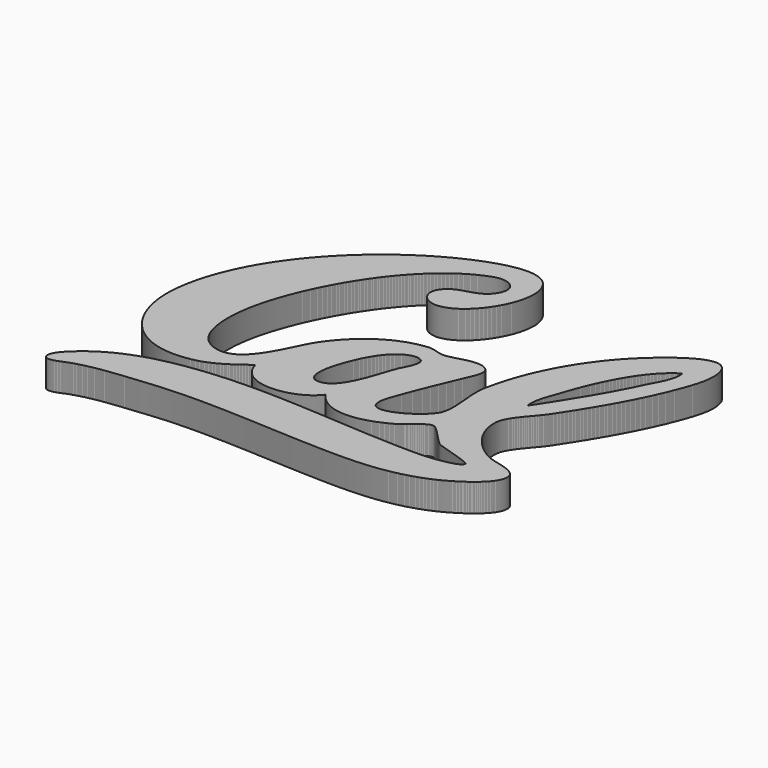
from build123d import *

# Parameters (mm, degrees)
F1_DEPTH = 3


# Not quite as in the source:
# - ends of sketch curves that miss each other by under 0.0002 mm in the source are joined


with BuildPart() as f1:
    # F0 (on Top) → F1 (new body)
    with BuildSketch(Plane.XY):
        Polygon((-8.5479254925, -6.1463442269), (-8.4652511503, -6.0838313976), (-8.4426561661, -6.1739883071), (-8.4180824511, -6.262318306), (-8.3915706833, -6.3488323978), (-8.363141104, -6.4335411935), (-8.3328444136, -6.5164661115), (-8.3006910272, -6.5975971292), (-8.2667214266, -6.6769554688), (-8.2309762901, -6.7545521337), (-8.1934658364, -6.8303873201), (-8.1542307438, -6.9044720314), (-8.1133114942, -6.9768274898), (-8.0707185025, -7.0474436727), (-8.0265024693, -7.1163419986), (-7.9806836357, -7.1835330783), (-7.9333028761, -7.2490176967), (-7.884370213, -7.3128062687), (-7.8339365432, -7.374909994), (-7.7820221077, -7.4353394834), (-7.7286675848, -7.4941057405), (-7.6738932155, -7.5512193764), (-7.6177398743, -7.6066811757), (-7.5602278022, -7.6605017497), (-7.5013976774, -7.7126921016), (-7.4412695448, -7.7632730613), (-7.379884475, -7.8122351948), (-7.3172729277, -7.8595893094), (-7.2534549477, -7.9053562347), (-7.188481628, -7.9495369519), (-7.1223629911, -7.9921418757), (-7.055139519, -8.0331922281), (-6.9868318452, -8.0726781831), (-6.9174908665, -8.1106109402), (-6.8471366278, -8.147011329), (-6.7757895662, -8.181879742), (-6.7035005786, -8.2152273789), (-6.6302897099, -8.2470750693), (-6.5561878121, -8.2774131831), (-6.4812253449, -8.3062525277), (-6.4054325716, -8.3336141289), (-6.3288503668, -8.3594987715), (-6.2514987753, -8.3839272852), (-6.173408649, -8.4068900399), (-6.0946204701, -8.4284082578), (-6.0151546758, -8.4484823312), (-5.9350415295, -8.467133286), (-5.8543217094, -8.4843721256), (-5.7730158491, -8.5001890239), (-5.6911644305, -8.5146052029), (-5.6087979134, -8.5276314698), (-5.5259365386, -8.5392784357), (-5.4426211807, -8.5495468854), (-5.3588718845, -8.5584576486), (-5.2747399393, -8.5660014876), (-5.1902351713, -8.5721990359), (-5.1053980625, -8.5770715156), (-5.0202596611, -8.580599078), (-4.9348498383, -8.5828231863), (-4.8491996422, -8.5837239918), (-4.7633289215, -8.5833325428), (-4.6772889655, -8.5816396017), (-4.5910998189, -8.5786659982), (-4.5047919415, -8.5744225395), (-4.4183957927, -8.5689200328), (-4.3319524434, -8.5621490443), (-4.2454715235, -8.5541404262), (-4.1590041261, -8.5448951594), (-4.0725706884, -8.5344136364), (-3.9862116925, -8.5227170791), (-3.8999473793, -8.5098160988), (-3.813808601, -8.4957010652), (-3.7278356434, -8.4804034192), (-3.6420489437, -8.4639235532), (-3.5564891801, -8.4462724705), (-3.4711870085, -8.4274507599), (-3.3861624738, -8.4074792509), (-3.3014564504, -8.3863587283), (-3.2170891792, -8.3640998034), (-3.1331013386, -8.3407134793), (-3.0495233883, -8.3162105635), (-2.9663859839, -8.2905916445), (-2.8837193891, -8.2638777481), (-2.8015542595, -8.2360694631), (-2.7199106401, -8.207187619), (-2.6388398201, -8.1772229783), (-2.5583516258, -8.1461961743), (-2.4784969539, -8.1141184068), (-2.3992962418, -8.0809900682), (-2.320779949, -8.0468219657), (-2.242978339, -8.0116351252), (-2.1659222639, -7.9754199166), (-2.0896520094, -7.9382077807), (-2.0141882091, -7.8999888912), (-1.9395613225, -7.8607740554), (-1.8658118317, -7.8205844953), (-1.792960174, -7.7794206034), (-1.721036809, -7.7372931868), (-1.650082611, -7.6942030305), (-1.5801276475, -7.6501813789), (-1.5111927479, -7.6052081872), (-1.4433181982, -7.559314896), (-1.3765244356, -7.5125018978), (-1.3108519421, -7.4647904146), (-1.2463315698, -7.4161708164), (-1.1829937783, -7.3666539105), (-1.1208586124, -7.3162605266), (-1.0599667504, -7.2650016679), (-1.0003490443, -7.2128677047), (-0.94204578, -7.1598900775), (-0.8850673723, -7.1060587639), (-0.8294543033, -7.0513949861), (-0.7752372287, -6.9958993325), (-0.7224464121, -6.9395928291), (-0.6711227279, -6.8824762607), (-0.6212761984, -6.8245600422), (-0.5729579168, -6.7658451545), (-0.5261877317, -6.7063626459), (-0.4809966913, -6.6460926678), (-0.4209650077, -6.7283853105), (-0.3599123803, -6.8084809824), (-0.2978588538, -6.8864005134), (-0.2348140584, -6.9621747555), (-0.1708086498, -7.0358042972), (-0.1058418433, -7.1073300131), (-0.0399444908, -7.1767422732), (0.0268739739, -7.244082148), (0.0945931134, -7.3093500301), (0.1632032979, -7.3725767716), (0.2326740676, -7.4337731795), (0.3029954003, -7.4929496688), (0.3741576658, -7.5501370915), (0.4461306007, -7.6053564734), (0.5189039865, -7.6586080108), (0.5924681932, -7.7099225558), (0.666792761, -7.7593109155), (0.7418678638, -7.8067937234), (0.8176836755, -7.8523916129), (0.8942097363, -7.8961153913), (0.9714261976, -7.9379961068), (1.0493330595, -7.9780337595), (1.1279102772, -8.0162491789), (1.2071277834, -8.0526736096), (1.2869857743, -8.0873172702), (1.3674537902, -8.1201909678), (1.4485119827, -8.1513257508), (1.5301603516, -8.1807216192), (1.6123688298, -8.2084098174), (1.695127591, -8.2344109789), (1.7784163943, -8.2587357146), (1.8622252172, -8.2813944395), (1.9465239925, -8.302418398), (2.0312924791, -8.321818201), (2.1165412882, -8.3396140898), (2.2022297414, -8.3558170676), (2.2883379902, -8.3704581827), (2.3748764493, -8.3835474576), (2.4617942219, -8.3950960919), (2.5491021153, -8.4051345453), (2.6367592549, -8.4136636025), (2.7247766443, -8.4207239419), (2.8131132127, -8.4263061296), (2.9017595263, -8.4304512363), (2.9906953442, -8.4331698731), (3.0799210588, -8.4344824771), (3.1693957955, -8.4343898332), (3.2591203393, -8.4329328159), (3.3490742529, -8.4301118176), (3.439227469, -8.4259580827), (3.5295799877, -8.4204716113), (3.6201119604, -8.4136834516), (3.7108033422, -8.4056144332), (3.8016236736, -8.3962753634), (3.8925833692, -8.3856762646), (3.9836421434, -8.3738485775), (4.0748003884, -8.3608127393), (4.1660274485, -8.3465693387), (4.2573239123, -8.3311490314), (4.3486491015, -8.3145628209), (4.4400034086, -8.2968311444), (4.5313565701, -8.2779750279), (4.6227087822, -8.2580046899), (4.7140297815, -8.2369411562), (4.8053097417, -8.2148050604), (4.8965388368, -8.1916170358), (4.9876761922, -8.1673778673), (5.0787225927, -8.1421284293), (5.1696678198, -8.1158689181), (5.2604715876, -8.0886307743), (5.3511338961, -8.0604139979), (5.4416451153, -8.0312494409), (5.5319647632, -8.0011583255), (5.6220928397, -7.9701406517), (5.7120096925, -7.9382376862), (5.8017051029, -7.9054496254), (5.891138589, -7.8717976913), (5.9803205654, -7.8372919062), (6.0692211613, -7.8019737333), (6.1578299618, -7.7658331501), (6.2461170958, -7.7289116199), (6.3340723448, -7.6912093386), (6.4216860787, -7.6527571585), (6.5089380566, -7.6135656905), (6.5957978187, -7.5736457419), (6.6822659538, -7.5330279684), (6.7683222208, -7.4917229813), (6.8539463787, -7.4497413914), (6.939118775, -7.4071244657), (7.023828995, -7.3638621817), (7.1080573862, -7.3199958064), (7.1917835115, -7.275525732), (7.2749873259, -7.2304727884), (7.3576694182, -7.1848676313), (7.4397991325, -7.1387108494), (7.5213566201, -7.0920334908), (7.6023418811, -7.0448355557), (7.6642986499, -7.0064466744), (7.7301681453, -6.9620741277), (7.7996840787, -6.9122239254), (7.8725803579, -6.8574122958), (7.948591087, -6.798165686), (8.0274497812, -6.734979887), (8.1088901521, -6.6683609086), (8.1926464999, -6.5988454164), (8.27845234, -6.5269292016), (8.3660517986, -6.4531282962), (8.4551683687, -6.3779489063), (8.5455461767, -6.3019070641), (8.636909108, -6.2255294126), (8.7289904817, -6.1493015244), (8.8215348166, -6.073759869), (8.914275628, -5.9994002374), (9.0069468237, -5.9267388581), (9.0992823114, -5.8562919593), (9.1910057803, -5.7885759656), (9.2818711829, -5.7240862759), (9.3715921861, -5.6633497294), (9.4599231347, -5.6068821621), (9.5465873255, -5.5551795614), (9.6313188625, -5.5087683743), (9.7138514573, -5.4681546104), (9.7939290399, -5.4338440834), (9.8712754958, -5.4063634365), (9.9456245365, -5.3862186793), (10.0167303107, -5.3739154292), (10.0843062891, -5.369970307), (10.1324731358, -5.3747086563), (10.1846279323, -5.3880287912), (10.240537236, -5.4094854091), (10.2999672118, -5.4386127704), (10.3627048542, -5.4749651801), (10.428526743, -5.5180869209), (10.497209458, -5.5675222754), (10.568519164, -5.6228055039), (10.6422428556, -5.6834909115), (10.7181468939, -5.749122977), (10.7960178812, -5.8192355684), (10.8756327896, -5.8933934054), (10.9567575877, -5.9711205298), (11.0391792701, -6.0519712466), (11.1226539795, -6.1354902309), (11.206988755, -6.2212109581), (11.2919401317, -6.3086985405), (11.3772842969, -6.3974768236), (11.4627982228, -6.4871105273), (11.5482580967, -6.577123497), (11.6334509131, -6.6670700378), (11.7181430331, -6.7564946286), (11.8021110366, -6.844941552), (11.8851316995, -6.9319653093), (11.9669812091, -7.0170897459), (12.0474363413, -7.0998693632), (12.126273676, -7.1798484438), (12.2032697927, -7.2565712703), (12.2782012714, -7.3295821255), (12.3508448879, -7.3984355106), (12.4209666109, -7.4626554672), (12.4883638499, -7.5218063229), (12.5527925512, -7.5754225341), (12.6140393168, -7.6230379687), (12.6718709004, -7.6642175427), (12.7260841226, -7.6984949278), (12.7643115256, -7.7190337025), (12.8119588588, -7.7414360819), (12.8685240368, -7.7656401498), (12.9334837519, -7.7915435079), (13.0063253074, -7.8190639992), (13.0865560515, -7.8480986368), (13.1736428504, -7.878565656), (13.2671032709, -7.9103618737), (13.3663941567, -7.9434159401), (13.4710330745, -7.9776246721), (13.5805073278, -8.0129059125), (13.6942833903, -8.0491574594), (13.8118792211, -8.0862965669), (13.9327614903, -8.1242312518), (14.0564377422, -8.1628687457), (14.1823952802, -8.2021268916), (14.3101107966, -8.2419032913), (14.439092032, -8.2821153951), (14.5688156788, -8.322660805), (14.6987692365, -8.3634675822), (14.8284600533, -8.4044327401), (14.9573549954, -8.4454745138), (15.0849614109, -8.4864899167), (15.2107667994, -8.52740701), (15.3342578757, -8.5681129808), (15.4549219431, -8.6085256719), (15.5722565236, -8.6485627301), (15.6857383095, -8.6881217569), (15.7948750415, -8.727120203), (15.8991436081, -8.7654658887), (15.9980311164, -8.8030664382), (16.0910348922, -8.8398292796), (16.177642239, -8.8756722556), (16.2573502862, -8.9104925757), (16.3296463372, -8.9442080828), (16.3940072806, -8.9767265971), (16.4499306383, -9.0079657655), (16.4969133438, -9.0378125785), (16.5344430927, -9.0662053164), (16.5619963813, -9.0930313623), (16.5790807539, -9.118197948), (16.5851837101, -9.141633135), (16.5774936365, -9.2069689263), (16.5528863558, -9.2691539344), (16.5129068409, -9.3282607183), (16.4590788427, -9.3843213546), (16.3929467457, -9.4373777464), (16.3160451079, -9.4874924301), (16.2299181175, -9.53469709), (16.1360897217, -9.5790340216), (16.0361046972, -9.620565565), (15.9314968174, -9.6593133823), (15.8238008366, -9.6953502284), (15.7145607468, -9.7286975691), (15.6053111062, -9.7594179409), (15.4975860805, -9.7875534429), (15.3929298578, -9.8131357595), (15.2928667777, -9.8362276233), (15.1989412246, -9.8568709374), (15.112687168, -9.8750975822), (15.0356493847, -9.890969898), (14.9693620404, -9.904529984), (14.9153591046, -9.9158097208), (14.8199892108, -9.9357652008), (14.7239781267, -9.9548027555), (14.6273266369, -9.9729632593), (14.5300655936, -9.9902563422), (14.4322156302, -10.0066918304), (14.3337977726, -10.0222999873), (14.234843069, -10.0371006617), (14.135361738, -10.0510936571), (14.0353852204, -10.0643192596), (13.9349237346, -10.0767772728), (13.8340187439, -10.0884975678), (13.7326804669, -10.0994799484), (13.6309303217, -10.1097751153), (13.5287987681, -10.1193722612), (13.4263066356, -10.1282914309), (13.3234749502, -10.1365628878), (13.2203245414, -10.1442066769), (13.1168758466, -10.1512224056), (13.0131500877, -10.157650556), (12.9091779207, -10.1634905394), (12.8049801751, -10.1687624008), (12.7005778769, -10.1734964035), (12.5960016817, -10.177691959), (12.4912523746, -10.1813899415), (12.38637083, -10.1845895665), (12.2813780736, -10.1873210972), (12.1762843242, -10.1895843374), (12.0711312409, -10.1914193769), (11.9659190201, -10.1928364342), (11.8606887324, -10.193844943), (11.7554612074, -10.1944649483), (11.6502472524, -10.1947269096), (11.545087938, -10.1946402608), (11.4399834605, -10.1942152204), (11.3349752829, -10.1934816594), (11.23007382, -10.1924496004), (11.1253000978, -10.1911493066), (11.0206949906, -10.1895799934), (10.9162590871, -10.1877723164), (10.8120336542, -10.1857459282), (10.708018888, -10.1835110473), (10.6042662742, -10.1810871299), (10.5007657901, -10.1784845909), (10.3975693139, -10.1757433237), (10.294687064, -10.172863132), (10.1921398701, -10.1698640608), (10.0899487581, -10.1667763733), (9.9881443838, -10.1635994811), (9.8867375545, -10.1603638436), (9.7857591222, -10.157079091), (9.6852403314, -10.1537752905), (9.5851811821, -10.150452442), (9.4856233335, -10.1471506352), (9.386587223, -10.1438694776), (9.2880834614, -10.1406292104), (9.1901432934, -10.1374599006), (9.0927973747, -10.1343609598), (8.9946229634, -10.1312370372), (8.8963644486, -10.127992061), (8.7980326377, -10.1246564907), (8.6996169195, -10.1212100852), (8.6011176866, -10.1176732819), (8.5025447651, -10.1140254473), (8.4038883288, -10.1102872148), (8.3051483777, -10.1064585844), (8.2063349342, -10.1025291413), (8.1074483908, -10.0985193228), (8.0084781363, -10.0944088877), (7.9094450006, -10.090217881), (7.81032835, -10.0859364764), (7.7111385994, -10.0815746963), (7.6118757489, -10.0771325407), (7.5125397984, -10.0726100097), (7.413130748, -10.0680071032), (7.3136485976, -10.0633238213), (7.2141035658, -10.0585599676), (7.1144858265, -10.0537361758), (7.0147949872, -10.0488320084), (6.915041659, -10.0438677066), (6.8152254494, -10.0388228332), (6.7153365323, -10.0337180215), (6.6153851262, -10.0285530753), (6.5153608164, -10.0233179723), (6.4152842363, -10.0180225386), (6.3151351448, -10.0126773853), (6.2149233682, -10.007261879), (6.1146492988, -10.0017964568), (6.0143231553, -9.9962809225), (5.9139245005, -9.9907156687), (5.8134735754, -9.9850900842), (5.7129605537, -9.9794248025), (5.612395458, -9.9737094087), (5.5117680695, -9.9679440991), (5.4110888031, -9.9621388961), (5.3103474401, -9.9562939959), (5.2095541993, -9.9504092022), (5.1086990582, -9.9444949299), (5.0078020615, -9.9385303494), (4.9068431645, -9.9325362903), (4.8058325859, -9.9265125564), (4.7047703255, -9.9204591477), (4.6036666021, -9.914375868), (4.5025009783, -9.9082631096), (4.4012940877, -9.9021306989), (4.3000355154, -9.8959686133), (4.1987254575, -9.8897870716), (4.0973741328, -9.8835858774), (3.9959713227, -9.8773652271), (3.8945272456, -9.8711249243), (3.7930420979, -9.8648751878), (3.6915056608, -9.8586162137), (3.5899279569, -9.8523375872), (3.4883091824, -9.8460495269), (3.3866495334, -9.8397622515), (3.2849488137, -9.8334655422), (3.1831968047, -9.8271595954), (3.0814141399, -9.8208542372), (2.9796008192, -9.8145494676), (2.8777366017, -9.8082558977), (2.7758415321, -9.8019526978), (2.6739057842, -9.7956605013), (2.5719393805, -9.7893688934), (2.4699322986, -9.783088289), (2.367894757, -9.7768184919), (2.2658267558, -9.7705595019), (2.1637182725, -9.764321734), (2.0615895482, -9.7580945772), (1.9594201457, -9.7518784238), (1.8572204797, -9.7456832963), (1.7549907465, -9.7395194132), (1.6527305537, -9.7333663373), (1.5504505122, -9.7272443098), (1.4481301849, -9.7211537229), (1.3457898128, -9.7150839656), (1.2434295921, -9.7090452566), (1.1410393042, -9.7030377921), (1.038618949, -9.697061572), (0.9361787453, -9.6911164002), (0.8337190853, -9.6852227139), (0.7312291619, -9.6793500535), (0.6287197823, -9.6735288785), (0.5261907503, -9.6677489704), (0.4236522846, -9.662010133), (0.321084144, -9.6563229773), (0.218496351, -9.6506770884), (0.1158891018, -9.6450826851), (0.0132726151, -9.639539571), (-0.0893633279, -9.6340479424), (-0.1920185308, -9.628618018), (-0.2946931899, -9.623239579), (-0.3973666718, -9.6179224517), (-0.5000698285, -9.6126570061), (-0.6027716117, -9.6074630908), (-0.7054928511, -9.6023206611), (-0.8082229357, -9.5972499578), (-0.9109618655, -9.592250981), (-1.0137200552, -9.5873137084), (-1.1164766753, -9.5824581846), (-1.2192423368, -9.5776641688), (-1.3220166472, -9.5729520981), (-1.4247998027, -9.5683117539), (-1.5275918035, -9.5637431363), (-1.6303820383, -9.5592664861), (-1.7331811184, -9.5548615625), (-1.8359784325, -9.5505486064), (-1.9387845919, -9.5463073768), (-2.0415887891, -9.5421683334), (-2.1444016353, -9.5381112351), (-2.2472129119, -9.5341358858), (-2.3500120077, -9.5302625264), (-2.4528195563, -9.5264813307), (-2.5556253391, -9.5227921026), (-2.6584291598, -9.5192050606), (-2.7612310183, -9.5157202048), (-2.8640311111, -9.5123273165), (-2.9668188269, -9.5090466367), (-3.0696047769, -9.5058579245), (-3.1723885685, -9.5027816171), (-3.2751599833, -9.4998175183), (-3.377929436, -9.4969556056), (-3.4806863156, -9.49421612), (-3.5834412332, -9.4915788206), (-3.686173359, -9.4890637522), (-3.7889033265, -9.4866610886), (-3.8916207209, -9.4843808521), (-3.9943255422, -9.4822230428), (-4.0970177905, -9.4801876607), (-4.1996976618, -9.4782644872), (-4.3023647638, -9.4764739594), (-4.4050190965, -9.4748160774), (-4.5076506374, -9.4732804264), (-4.6102692129, -9.4718876398), (-4.7128649966, -9.4706170842), (-4.8154480111, -9.4694791744), (-4.9180078413, -9.4684839327), (-5.0205547061, -9.4676315555), (-5.1230785829, -9.4669116279), (-5.2255792757, -9.4663343684), (-5.3280670028, -9.4658999734), (-5.4305213273, -9.4656080504), (-5.5329522714, -9.4654690141), (-5.6353700537, -9.4654830609), (-5.7377544334, -9.4656395797), (-5.8401154326, -9.4659489853), (-5.9424528554, -9.4664214963), (-6.0447568753, -9.4670364793), (-6.1470373188, -9.4678145678), (-6.249283967, -9.4687555655), (-6.3515070387, -9.4698596686), (-6.4537065339, -9.4711268771), (-6.5558620153, -9.4725567987), (-6.6579939201, -9.4741498256), (-6.7600918336, -9.4759159804), (-6.8621559519, -9.4778450445), (-6.9641858826, -9.479957455), (-7.0661820181, -9.4822327747), (-7.1681439661, -9.4846914409), (-7.2700719227, -9.4873232349), (-7.3719554731, -9.4901381791), (-7.4738152507, -9.4931264474), (-7.5756202074, -9.4963078884), (-7.6774013912, -9.4996626534), (-7.7791277541, -9.503210591), (-7.880830148, -9.5069420713), (-7.9824777208, -9.5108667243), (-8.0840909099, -9.5149849423), (-8.1856594966, -9.5192965292), (-8.2871834809, -9.523801485), (-8.3886628628, -9.5284998096), (-8.490097446, -9.5334017217), (-8.5914872307, -9.5385072212), (-8.6928324129, -9.5438060897), (-8.7941326004, -9.5493187642), (-8.8953777706, -9.55503483), (-8.9965781422, -9.5609544832), (-9.0977234966, -9.5670775278), (-9.1988236599, -9.573424597), (-9.2998790246, -9.5799752537), (-9.4008789797, -9.586749739), (-9.5018239176, -9.5937276154), (-9.6027132496, -9.600939539), (-9.7035473682, -9.6083650725), (-9.804336492, -9.6160044121), (-9.9050597913, -9.6238776026), (-10.0057378996, -9.6319748178), (-10.1063503797, -9.6402956653), (-10.20690745, -9.6488403412), (-10.3074087184, -9.657629283), (-10.4078443585, -9.666641857), (-10.5082243927, -9.6758884781), (-10.6085488211, -9.6853691463), (-10.7088072288, -9.6950938841), (-10.8089998121, -9.7050524727), (-10.9091365933, -9.7152553271), (-11.0091971352, -9.7257020548), (-11.109201875, -9.7363930483), (-11.2091506166, -9.7473385261), (-11.3090231189, -9.7585278772), (-11.4088296006, -9.7699612978), (-11.5085698654, -9.7816490066), (-11.6082439132, -9.7935910035), (-11.7078415256, -9.8057870923), (-11.8073727249, -9.8182476879), (-11.9068377074, -9.8309625716), (-12.0062362767, -9.8439419621), (-12.1055481919, -9.8571752483), (-12.2048037165, -9.8706834561), (-12.303972587, -9.8844455595), (-12.4030748481, -9.8984823884), (-12.5021002814, -9.9127937464), (-12.6010490829, -9.927369415), (-12.6999208603, -9.9422298314), (-12.7987160061, -9.9573545583), (-12.8974343239, -9.9727538143), (-12.9960756176, -9.9884378182), (-13.0946398872, -10.0044065698), (-13.1931171103, -10.0206496543), (-13.2915173092, -10.0371774867), (-13.3898402879, -10.0540002854), (-13.48807622, -10.0710974171), (-13.5862245169, -10.0884995376), (-13.684295986, -10.1061761872), (-13.7822798199, -10.1241578257), (-13.8801764111, -10.1424240157), (-13.9779955857, -10.1609953907), (-14.0757171028, -10.1798613397), (-14.1733612034, -10.1990324737), (-14.2709076464, -10.2184981817), (-14.3683766729, -10.2382690747), (-14.4657478456, -10.2583447603), (-14.5630209684, -10.2787354571), (-14.6602166746, -10.2994313389), (-14.757314527, -10.3204320132), (-14.8543143295, -10.3417476988), (-14.9512263007, -10.3633785919), (-15.0480504405, -10.3853246923), (-15.1447661155, -10.4075958263), (-15.2413939591, -10.4301821678), (-15.3379237528, -10.4530835204), (-15.4343553003, -10.4763101029), (-15.5324269593, -10.500365523), (-15.6304280848, -10.5249000408), (-15.7283685031, -10.5499342897), (-15.8262177546, -10.5754574624), (-15.9239960802, -10.6014801701), (-16.0216828465, -10.6280122388), (-16.119268031, -10.6550432539), (-16.2167412191, -10.6825832376), (-16.314112433, -10.7106426048), (-16.4113612356, -10.7392209632), (-16.5084876269, -10.7683183126), (-16.6054711695, -10.7979342608), (-16.7023216898, -10.828089441), (-16.7990291653, -10.8587734386), (-16.8955731588, -10.889985861), (-16.9919532779, -10.9217471456), (-17.0881695225, -10.9540572922), (-17.1842118703, -10.9869058862), (-17.2800594916, -11.0203129722), (-17.3757330199, -11.0542687242), (-17.4711913844, -11.0887825759), (-17.5664548263, -11.1238651383), (-17.661513323, -11.1595059966), (-17.7563358264, -11.1957249994), (-17.8509429699, -11.2325123205), (-17.9453139238, -11.2698880047), (-18.0394490805, -11.3078316148), (-18.1333378291, -11.3463633919), (-18.2269597322, -11.3854829434), (-18.320335031, -11.4252008805), (-18.4134330695, -11.4655166145), (-18.506254044, -11.5064199267), (-18.5987973658, -11.5479414732), (-18.6910429902, -11.5900604241), (-18.7830007433, -11.6327974129), (-18.8746401655, -11.6761416325), (-18.9659814978, -11.7201036937), (-19.0569938882, -11.7646932267), (-19.1476875552, -11.8099104276), (-19.2380522804, -11.8557551003), (-19.3280676263, -11.9022268522), (-19.4177434193, -11.9493463169), (-19.5070594183, -11.9971028832), (-19.5960154271, -12.04550677), (-19.6846012271, -12.0945577808), (-19.7728065997, -12.1442557195), (-19.8606415672, -12.194611001), (-19.9480754739, -12.2456230366), (-20.035118146, -12.2973124597), (-20.1217597571, -12.349658637), (-20.207979674, -12.4026713946), (-20.2937877227, -12.4563713659), (-20.3791740772, -12.5107379175), (-20.4641179077, -12.5657910943), (-20.5486294328, -12.6215310924), (-20.632698434, -12.6779577156), (-20.7163042779, -12.7350807901), (-20.7994469643, -12.792900316), (-20.8821264934, -12.8514162932), (-20.9643324502, -12.9106387442), (-21.04605442, -12.9705776913), (-21.1272825766, -13.0312125011), (-21.2080163313, -13.0925738294), (-21.2882456618, -13.1546512615), (-21.3679703718, -13.2174550159), (-21.4471700241, -13.2809847003), (-21.5258444225, -13.3452505332), (-21.6039937632, -13.410242296), (-21.6815974127, -13.4759698149), (-21.7586551749, -13.5424433087), (-21.8351568311, -13.6096625809), (-21.9110921628, -13.6776274355), (-21.9623559847, -13.724019575), (-22.0182552603, -13.7749576786), (-22.0782122377, -13.8301853158), (-22.1416697982, -13.8894362297), (-22.2080295563, -13.9524638159), (-22.2767243708, -14.0189914029), (-22.3471660749, -14.0887725823), (-22.4187977461, -14.1615308789), (-22.4910310213, -14.2370301031), (-22.5632987594, -14.3149935832), (-22.6350027712, -14.3951644963), (-22.7055857417, -14.4772868041), (-22.7744494815, -14.5611036837), (-22.8410470908, -14.6463490745), (-22.9047803802, -14.7327661534), (-22.9650717936, -14.8200882713), (-23.0213537978, -14.9080591938), (-23.0730484444, -14.9964327089), (-23.119568155, -15.0849317525), (-23.1603556149, -15.1733002866), (-23.1948126347, -15.261281488), (-23.2223716809, -15.3486191225), (-23.2424551977, -15.4350465407), (-23.2544854329, -15.5203073122), (-23.2578950493, -15.6041349838), (-23.2520856613, -15.6862829513), (-23.2365001503, -15.7664849578), (-23.2105507418, -15.8444741579), (-23.1756644848, -15.9130098383), (-23.1319737813, -15.9705202943), (-23.0800903908, -16.0176203928), (-23.0206571207, -16.0549051523), (-22.9542861228, -16.0829690023), (-22.881630227, -16.1024173761), (-22.8032915627, -16.1138342886), (-22.7199125449, -16.1178351954), (-22.6321053253, -16.1150145262), (-22.5405229303, -16.1059674955), (-22.4457674889, -16.0912781183), (-22.3484812203, -16.0715720687), (-22.2492764722, -16.0474335579), (-22.1488062709, -16.0194578004), (-22.0476723533, -15.9882492484), (-21.9465175269, -15.9544029202), (-21.8459639658, -15.9185236603), (-21.7466342366, -15.881195876), (-21.6491707544, -15.8430350231), (-21.5541858671, -15.8046253124), (-21.4623119674, -15.7665717849), (-21.3741814482, -15.7294794813), (-21.2904168758, -15.6939328088), (-21.2116404245, -15.6605366121), (-21.1384947056, -15.6298961281), (-21.0715920669, -15.6025955679), (-21.01157512, -15.5792401685), (-20.9590457977, -15.5604241633), (-20.8607205784, -15.527746406), (-20.7622988945, -15.4958334752), (-20.6638013797, -15.4646755447), (-20.5652282299, -15.4342623958), (-20.466569423, -15.4045836138), (-20.3678355698, -15.3756189577), (-20.269016648, -15.3473580125), (-20.1701334873, -15.3197807335), (-20.0711656503, -15.2928867283), (-19.9721237481, -15.2666557559), (-19.8730181956, -15.2410777938), (-19.773828948, -15.2161320124), (-19.6745764424, -15.1918188041), (-19.5752408302, -15.1681071206), (-19.4758425488, -15.1449973544), (-19.3763819904, -15.1224690683), (-19.2768387179, -15.1005218697), (-19.177244172, -15.079115473), (-19.0775673043, -15.0582697266), (-18.9778395556, -15.0379443448), (-18.8780404886, -15.0181389352), (-18.7781702996, -14.998843279), (-18.6782498181, -14.9800373316), (-18.5782588032, -14.9617104818), (-18.4782076697, -14.9438527073), (-18.3780970062, -14.9264333522), (-18.2779368351, -14.9094628314), (-18.1777071115, -14.8929203151), (-18.0774184467, -14.8767855625), (-17.9770812552, -14.861048551), (-17.8766855148, -14.8456988658), (-17.7762316179, -14.8307160698), (-17.675729783, -14.816100359), (-17.575170184, -14.8018311002), (-17.4745634319, -14.7878880522), (-17.3738993081, -14.7742710189), (-17.2731886198, -14.7609495406), (-17.1724311709, -14.7479338359), (-17.0716173312, -14.7351930528), (-16.9707677343, -14.7227173651), (-16.8698621392, -14.7104961617), (-16.7689111568, -14.6985092016), (-16.6679250058, -14.6867566811), (-16.5668836413, -14.6752177705), (-16.4658078931, -14.6638724249), (-16.3646875425, -14.6527204482), (-16.2635229819, -14.6417414031), (-16.1623146037, -14.6309148524), (-16.0610726266, -14.6202409923), (-15.9597972467, -14.6097096042), (-15.858478834, -14.5992898361), (-15.7571175849, -14.5889714693), (-15.6557339364, -14.5787548962), (-15.5543078438, -14.5686192872), (-15.4528497219, -14.5585546199), (-15.3513497445, -14.5485402608), (-15.2498285451, -14.5385663838), (-15.1482761011, -14.528622574), (-15.046692609, -14.5186986128), (-14.9450784609, -14.508774063), (-14.8434340495, -14.4988284873), (-14.7417593746, -14.4888618858), (-14.6400648511, -14.4788642361), (-14.538340849, -14.468804686), (-14.4365871721, -14.4586934542), (-14.3348148238, -14.4484898624), (-14.233023608, -14.4382041294), (-14.1312036984, -14.4278156215), (-14.029365706, -14.4173040979), (-13.9275098271, -14.4066593398), (-13.8256258431, -14.3958811511), (-13.7237247573, -14.3849288535), (-13.6236078089, -14.3742254832), (-13.5234146212, -14.3637659862), (-13.423155609, -14.3535403401), (-13.32283038, -14.3435689821), (-13.2224293041, -14.3338210602), (-13.1219622075, -14.3243172078), (-13.0214294827, -14.3150369878), (-12.9208307371, -14.3060008372), (-12.8201663634, -14.2971883189), (-12.7194361651, -14.2886096516), (-12.6186403387, -14.2802546165), (-12.5177891025, -14.27212341), (-12.4168722381, -14.2642158357), (-12.3158899417, -14.2565216751), (-12.2148522356, -14.249051343), (-12.1137489013, -14.2418046432), (-12.0126005722, -14.2347717495), (-11.9113767886, -14.2279418546), (-11.8101080102, -14.2213257659), (-11.7087737997, -14.2149230908), (-11.6073945944, -14.2087342218), (-11.5059503495, -14.2027383292), (-11.4044611098, -14.1969562428), (-11.302917049, -14.1913673289), (-11.201317971, -14.1859818064), (-11.0996638758, -14.1807996751), (-10.9979653744, -14.1758006941), (-10.8962118558, -14.1710051044), (-10.7944137348, -14.1664028835), (-10.692560989, -14.1619836166), (-10.5906636407, -14.1577577186), (-10.4887218863, -14.1537149709), (-10.3867355294, -14.149865592), (-10.2847049626, -14.1461891447), (-10.1826299896, -14.1426958477), (-10.0805106104, -14.139385701), (-9.9783470212, -14.1362484858), (-9.876139222, -14.1332842023), (-9.7738972352, -14.1305032653), (-9.6716112347, -14.1278850412), (-9.5692812204, -14.1254295302), (-9.4669170185, -14.1231573657), (-9.3645192176, -14.1210378917), (-9.2620772067, -14.1190913494), (-9.1596015969, -14.1172974976), (-9.057092192, -14.1156665551), (-8.9545489918, -14.1141985219), (-8.8519721927, -14.1128831792), (-8.7493617947, -14.1117205271), (-8.6467177976, -14.1107105657), (-8.5440504203, -14.109853491), (-8.4413394216, -14.1091386922), (-8.3386050425, -14.1085767801), (-8.2358474793, -14.1081575363), (-8.1330565134, -14.1078807645), (-8.0302423633, -14.1077466608), (-7.9273950067, -14.1077448105), (-7.8245244659, -14.1078856285), (-7.7216309372, -14.108158896), (-7.6187144206, -14.1085646131), (-7.5157749161, -14.1091027797), (-7.4128124236, -14.109773396), (-7.3098271394, -14.1105662432), (-7.2068188673, -14.11149154), (-7.1037980221, -14.112539264), (-7.0007545813, -14.1136990004), (-6.8976983713, -14.1149913825), (-6.7946093471, -14.1163955808), (-6.6915181647, -14.1179121838), (-6.5884041905, -14.1195510179), (-6.4852780356, -14.1212918418), (-6.3821393076, -14.123155093), (-6.278988399, -14.1251203341), (-6.1758253096, -14.1271875651), (-6.0726396248, -14.1293668085), (-5.9694519778, -14.131648238), (-5.8662521502, -14.1340316575), (-5.7630505567, -14.1365070445), (-5.6598265639, -14.1390842253), (-5.5566110239, -14.1417535698), (-5.4533732807, -14.1445144894), (-5.3501439903, -14.1473675728), (-5.2468924969, -14.1503122313), (-5.1436494561, -14.1533490535), (-5.0404048457, -14.1564676247), (-4.937148447, -14.1596677486), (-4.8338904787, -14.1629496214), (-4.7306411593, -14.1663134393), (-4.6273800516, -14.16975881), (-4.5241277891, -14.1732759071), (-4.4208741532, -14.1768645346), (-4.3176191438, -14.1805246924), (-4.2143729796, -14.1842565767), (-4.1111254419, -14.1880599913), (-4.0078867493, -14.1919351324), (-3.9046470758, -14.1958613666), (-3.8014162474, -14.1998593273), (-3.6981944604, -14.2039187959), (-3.5949819109, -14.2080295537), (-3.4917784028, -14.2122018195), (-3.3885839361, -14.2164355932), (-3.2853989032, -14.2207104376), (-3.1822229116, -14.2250467898), (-3.0790563539, -14.2294242127), (-2.9759092523, -14.2338531212), (-2.8727713883, -14.2383333189), (-2.7696533729, -14.2428445648), (-2.6665445951, -14.2474071001), (-2.5634554697, -14.2520109022), (-2.4603759743, -14.2566455563), (-2.3573161313, -14.2613214774), (-2.2542863555, -14.2660286429), (-2.1512662097, -14.2707666605), (-2.0482659125, -14.2755357263), (-1.9452854639, -14.2803358404), (-1.8423248639, -14.2851670027), (-1.7393945274, -14.2900191909), (-1.6364842357, -14.2948922088), (-1.5335939888, -14.2997860563), (-1.4307342015, -14.304690711), (-1.3278942628, -14.309626414), (-1.2250847838, -14.3145729243), (-1.1223057644, -14.3195302417), (-1.019546986, -14.3244981702), (-0.9168288859, -14.3294771022), (-0.8141312231, -14.3344564265), (-0.7114638236, -14.3394567767), (-0.6088272762, -14.344447497), (-0.5062314071, -14.3494492206), (-0.40366639, -14.3544413143), (-0.3011320287, -14.3594339966), (-0.1986283233, -14.3644272675), (-0.0961656886, -14.3694111046), (0.0062662903, -14.3743955304), (0.1086570023, -14.3793603037), (0.2110066436, -14.3843156433), (0.3133254329, -14.3892613529), (0.4156029553, -14.39418741), (0.5178289922, -14.399094011), (0.6200241771, -14.403990982), (0.7221778989, -14.408858082), (0.8242903538, -14.4137055295), (0.926351127, -14.4185233023), (1.0283706333, -14.4233214227), (1.1303486765, -14.428089672), (1.2322750381, -14.4328282465), (1.3341597403, -14.4375267314), (1.4359927609, -14.4421955415), (1.5377843184, -14.4468344806), (1.6395238017, -14.4514233076), (1.7412116034, -14.4559824599), (1.8428473309, -14.4604915001), (1.9444311806, -14.4649606468), (2.0459629561, -14.4693796816), (2.1474428537, -14.4737588229), (2.2488604586, -14.4780880483), (2.3502360118, -14.4823567469), (2.4515492722, -14.4865755297), (2.55280024, -14.4907443967), (2.654009156, -14.4948527367), (2.7551453645, -14.4989011386), (2.8562293026, -14.5028892098), (2.9572507518, -14.5068171465), (3.0582197345, -14.510674534), (3.1591160096, -14.5144719832), (3.2599494034, -14.5181888608), (3.3607305269, -14.5218454077), (3.4614387466, -14.5254317977), (3.5620840849, -14.5289376161), (3.6626665419, -14.5323628628), (3.7631863138, -14.5357177564), (3.8636329857, -14.5389922746), (3.96401658, -14.5421760024), (4.0647880893, -14.5453318372), (4.165589862, -14.5484666461), (4.2664116795, -14.5515806253), (4.3672533457, -14.5546635563), (4.4681146642, -14.5577052204), (4.5690058538, -14.5607054214), (4.6699064772, -14.5636645518), (4.7708161419, -14.5665621743), (4.8717554814, -14.569408115), (4.9726936437, -14.5721927441), (5.0736608922, -14.5748950356), (5.1746269634, -14.5775360155), (5.2756014874, -14.5800848316), (5.3765948789, -14.5825515063), (5.4775865046, -14.5849262135), (5.5785863868, -14.5871985384), (5.6795947218, -14.5893786995), (5.7806007023, -14.5914362372), (5.8816149393, -14.5933913926), (5.9826266256, -14.5952137059), (6.0836359575, -14.5969133959), (6.1846429348, -14.5984904625), (6.2856573839, -14.5999242723), (6.3866588674, -14.6012152177), (6.4876471892, -14.60235308), (6.5886427865, -14.6033374669), (6.6896252221, -14.6041687708), (6.7905941036, -14.6048265545), (6.8915496271, -14.6053210365), (6.9925016189, -14.6056315834), (7.0934298379, -14.6057688063), (7.194354329, -14.6057118754), (7.2952546549, -14.6054611834), (7.396140838, -14.6050063152), (7.497002856, -14.6043576857), (7.5978503388, -14.6034844429), (7.6986734602, -14.6024072202), (7.7994820464, -14.6011053842), (7.9002556603, -14.5995793273), (8.0010143465, -14.5978082198), (8.1017380603, -14.5958128914), (8.2024364317, -14.59356249), (8.3031096569, -14.5910672343), (8.4037473211, -14.5883171018), (8.504349228, -14.585301874), (8.6049255963, -14.5820213545), (8.7054660112, -14.5784655211), (8.8059704726, -14.5746343737), (8.9064387843, -14.5705176936), (9.0068709464, -14.566115481), (9.107256544, -14.5614177133), (9.2076055996, -14.5564139759), (9.3079183093, -14.5511144872), (9.4081736473, -14.5454889838), (9.5083924432, -14.5395575106), (9.608564086, -14.5332998265), (9.7086885757, -14.5267159316), (9.8087657161, -14.5197956072), (9.908795311, -14.5125286347), (10.008767338, -14.504925429), (10.1086916232, -14.4969653565), (10.2085579481, -14.4886486136), (10.3083763351, -14.4799647853), (10.4081367617, -14.4709242865), (10.5078284208, -14.4614966576), (10.6074721419, -14.4517019434), (10.7070470955, -14.441520099), (10.8065735225, -14.4309405135), (10.9060207671, -14.4199637754), (11.0054194852, -14.4085892961), (11.1047388247, -14.3968074457), (11.2039992228, -14.3846178317), (11.3031900684, -14.3720002132), (11.4023115579, -14.3589648086), (11.5013632988, -14.3454911808), (11.6003352687, -14.3315897446), (11.6992475123, -14.3172396704), (11.7980695701, -14.3024517654), (11.8968317055, -14.2872050038), (11.9955032627, -14.2714999741), (12.0941046788, -14.2553362839), (12.1926253428, -14.2386936923), (12.2910552324, -14.2215826141), (12.3894145886, -14.2039924382), (12.4876827778, -14.1859133384), (12.5858698226, -14.1673348999), (12.6839759192, -14.1482673413), (12.7819802378, -14.1286906179), (12.879903412, -14.1086145557), (12.9777450492, -14.0880187176), (13.0754845162, -14.0668932774), (13.1731324238, -14.045258476), (13.2706881836, -14.0230836578), (13.3681415768, -14.0003690187), (13.465502822, -13.9771143627), (13.5627717232, -13.9533094712), (13.6599380616, -13.9289545403), (13.7570016411, -13.9040393514), (13.8539622654, -13.8785536859), (13.9508201308, -13.8525077625), (14.0475746486, -13.8258709252), (14.1442262112, -13.7986636114), (14.2407642077, -13.7708655799), (14.3371988566, -13.7424766346), (14.4335195469, -13.7134765345), (14.5297368896, -13.6838855205), (14.6258400776, -13.6536731331), (14.7218190883, -13.622849787), (14.8176941628, -13.5914048713), (14.9134448639, -13.5593387784), (15.0090810177, -13.5266308747), (15.1046028206, -13.493291379), (15.1999996614, -13.4593000501), (15.295281955, -13.4246669106), (15.3904390903, -13.3893717194), (15.4854712636, -13.353424695), (15.5803678639, -13.3168055966), (15.6751493282, -13.2795140316), (15.7698052419, -13.2415399777), (15.8643253864, -13.202883631), (15.9587097615, -13.1635449916), (16.0529681936, -13.123503426), (16.1471008788, -13.0827691529), (16.2410869874, -13.0413221273), (16.334947153, -12.9991721757), (16.4286605459, -12.956299253), (16.5222476033, -12.9127029669), (16.6156876917, -12.8683734912), (16.7089910298, -12.8233106297), (16.7640607081, -12.7962474963), (16.8218759059, -12.7673631741), (16.8823348294, -12.7366800622), (16.9453056177, -12.7042518046), (17.0106660398, -12.670101193), (17.0783144982, -12.6342608451), (17.1481291543, -12.5967739901), (17.2199775586, -12.5576636158), (17.2937581134, -12.5169623401), (17.3693489804, -12.474713392), (17.4466383432, -12.4309495857), (17.5254937523, -12.385693909), (17.6058136103, -12.3389789799), (17.687466056, -12.2908584421), (17.7703490997, -12.2413444763), (17.854330684, -12.1904805078), (17.939298993, -12.1382993505), (18.0251422104, -12.0848338188), (18.1117280828, -12.030117119), (18.1989550127, -11.9741818691), (18.2867009654, -11.9170610794), (18.3748439061, -11.8587877604), (18.4632619962, -11.7994051408), (18.551853442, -11.7389356201), (18.6404859902, -11.6774124048), (18.7290582393, -11.6148783314), (18.8174277175, -11.5513668027), (18.9055028495, -11.4869000217), (18.9931513821, -11.4215111951), (19.0802516728, -11.3552537703), (19.1667017318, -11.288139928), (19.2523693056, -11.2202028749), (19.3371531891, -11.151495666), (19.4209209327, -11.0820412893), (19.5035505018, -11.0118727551), (19.5849401025, -10.9410124628), (19.6649680924, -10.8695138598), (19.7435224594, -10.7973995417), (19.8204709498, -10.7247027151), (19.8957019439, -10.6514664126), (19.9690932107, -10.5777134261), (20.0405431526, -10.5034763734), (20.1099197125, -10.4287986796), (20.1771108779, -10.3537029404), (20.2419948105, -10.2782323846), (20.3044596939, -10.2024198264), (20.3643832972, -10.1262880575), (20.421643782, -10.0498803068), (20.4761395506, -9.9732291923), (20.5277485682, -9.8963677242), (20.5763385816, -9.8193291093), (20.6217977746, -9.7421461614), (20.6640245496, -9.6648514987), (20.7028764346, -9.5874785238), (20.7382620508, -9.5100596585), (20.7700391223, -9.4326385241), (20.7981058555, -9.3552375199), (20.8223402154, -9.2778896563), (20.8426305823, -9.200637966), (20.8588445065, -9.1235054369), (20.8708805867, -9.0465349056), (20.8786063733, -8.9697493599), (20.8819204651, -8.8931916365), (20.8806906085, -8.8168949419), (20.8748152061, -8.7408918939), (20.8641618083, -8.6652054806), (20.8486187952, -8.5898787346), (20.8262562852, -8.5128940127), (20.7971376058, -8.4391466202), (20.7615469163, -8.3685288771), (20.719788813, -8.3009327112), (20.672158066, -8.2362706833), (20.6189490532, -8.1744349175), (20.5604663709, -8.1153173412), (20.4969945707, -8.0588307118), (20.4288482714, -8.004856542), (20.3563118283, -7.9532973706), (20.2797004489, -7.9040653661), (20.1992979, -7.8570324115), (20.1153991478, -7.8121212862), (20.0283190074, -7.7692237218), (19.9383314194, -7.7282322346), (19.8457614173, -7.6890383596), (19.7508833341, -7.6515550505), (19.6540119849, -7.6156740386), (19.5554419435, -7.5812976663), (19.4554571729, -7.5483080351), (19.3543730768, -7.5166275323), (19.2524838367, -7.486138063), (19.150073808, -7.4567421659), (19.0474578057, -7.4283315725), (18.9449305999, -7.4008188438), (18.8427863723, -7.374085885), (18.7413196967, -7.3480350385), (18.6408353659, -7.3225684506), (18.5416279537, -7.2975884638), (18.4440020566, -7.2729870056), (18.3482420299, -7.2486666148), (18.2546522738, -7.2245090003), (18.1635379732, -7.2004367456), (18.0751933099, -7.1763317559), (17.9899026391, -7.1520965699), (17.9079909944, -7.1276227227), (17.8297327088, -7.1028231679), (17.7554321824, -7.0775796145), (17.6853841856, -7.0518046235), (17.6199033369, -7.0253797077), (17.5391372786, -6.9902934758), (17.4583801128, -6.9535408246), (17.3776733029, -6.9151516254), (17.2970478969, -6.8751457267), (17.2165353355, -6.8335634143), (17.1361766895, -6.7904141221), (17.0559927885, -6.7457178948), (16.9760355104, -6.6995146258), (16.8963252924, -6.6518039228), (16.8168935752, -6.6026260716), (16.7377920405, -6.552010747), (16.6590411255, -6.4999575566), (16.5806824895, -6.4465065899), (16.5027471808, -6.3916776958), (16.4252766625, -6.335500745), (16.3482813494, -6.2779857601), (16.2718233379, -6.2191724382), (16.1959230654, -6.159060387), (16.1206223873, -6.0976999147), (16.0459519595, -6.0350904327), (15.9719330041, -5.971272423), (15.8986272251, -5.9062651455), (15.8260452335, -5.8400888415), (15.7542282963, -5.7727631631), (15.6832078542, -5.7043283963), (15.6130350001, -5.63478356), (15.5437207377, -5.5641693326), (15.4753165522, -5.4925051701), (15.4078432734, -5.4198111174), (15.3413525831, -5.3461168493), (15.2758651145, -5.271432192), (15.2114123084, -5.1957974313), (15.1480352355, -5.1192220011), (15.0857755551, -5.0417459909), (15.0246537044, -4.9633690084), (14.9647115388, -4.8841413617), (14.9059797143, -4.8040624623), (14.8484896715, -4.7231725961), (14.7922926997, -4.6414810005), (14.7373996061, -4.5590181352), (14.6838620725, -4.4758136751), (14.631711147, -4.3918874687), (14.5809674632, -4.3072493423), (14.5316828989, -4.2219391892), (14.4838885024, -4.1359768581), (14.4376153219, -4.0493821975), (14.392894602, -3.9621852748), (14.3497571947, -3.8743957199), (14.3082547816, -3.7860432076), (14.2683981701, -3.6971581975), (14.2302388455, -3.6077601459), (14.1938078562, -3.5178689013), (14.1591464691, -3.4275041161), (14.1262656876, -3.3367064687), (14.0952268233, -3.2454747817), (14.066041076, -3.1538599521), (14.0387595387, -3.0618609987), (14.0134134558, -2.9695079888), (13.9900240495, -2.8768414045), (13.9686424128, -2.7838602648), (13.9492997902, -2.6905946367), (13.9320172076, -2.5970747839), (13.9168461503, -2.5033201624), (13.903817863, -2.4093608395), (13.892952979, -2.3152066414), (13.8842931576, -2.2208976577), (13.8778792733, -2.1264331037), (13.8737429629, -2.0318634836), (13.8719150786, -1.9371984277), (13.8724266686, -1.8424577843), (13.8753191959, -1.7476714247), (13.8806339275, -1.6528590011), (13.8883814743, -1.5580407546), (13.8986237368, -1.4632461637), (13.9101530382, -1.3854369053), (13.9259052101, -1.3066163268), (13.9457181281, -1.2268590978), (13.9694497127, -1.1462190584), (13.9969374469, -1.0647504408), (14.0280186178, -0.982497259), (14.0625515382, -0.8995337901), (14.1003632765, -0.8159042441), (14.1413221679, -0.7316724834), (14.1852450622, -0.6468829141), (14.2320002947, -0.5615993988), (14.2814151299, -0.4758763659), (14.3333474882, -0.3897676555), (14.3876348528, -0.3033274999), (14.4441251218, -0.216620154), (14.5026658007, -0.1296894353), (14.5630845466, -0.0426102097), (14.625249106, 0.0445843163), (14.6889869397, 0.1318294955), (14.7541559683, 0.2190714879), (14.8205836523, 0.3062456462), (14.8881379348, 0.3933085454), (14.9566360578, 0.480195342), (15.0259461604, 0.5668523922), (15.0959057257, 0.6532254636), (15.1663522371, 0.7392603238), (15.2371335924, 0.8248927181), (15.3080972973, 0.9100788288), (15.3790912498, 0.9947544012), (15.4499527369, 1.0788754215), (15.5205298528, 1.1623674162), (15.5906699069, 1.2451967864), (15.6602005563, 1.3272886662), (15.7289899398, 1.4085894119), (15.7968753446, 1.4890550098), (15.8636944499, 1.5686210087), (15.9293051764, 1.6472335688), (15.9935347884, 1.7248382613), (16.0562309879, 1.8013810502), (16.1172518914, 1.8767978768), (16.1764349821, 1.9510345088), (16.2336175471, 2.0240469323), (16.288657703, 2.0957710887), (16.3413929329, 2.1661527457), (16.3916607201, 2.2351376709), (16.4393191811, 2.3026618057), (16.484205603, 2.3686811362), (16.5405405673, 2.4533614683), (16.5968328914, 2.5381329832), (16.6530623341, 2.6229850697), (16.709239114, 2.7079179241), (16.7653528164, 2.7929415688), (16.8214036374, 2.8780457852), (16.8773913809, 2.9632407919), (16.9333060244, 3.048516174), (16.989167809, 3.1338825427), (17.044946275, 3.2193290906), (17.1006616634, 3.3048664288), (17.1562937332, 3.3904839462), (17.2118525069, 3.4761920578), (17.2673277658, 3.5619905672), (17.3227299247, 3.6478694521), (17.3780385464, 3.7338283201), (17.4332736757, 3.8198880007), (17.4884152679, 3.9060276644), (17.5434633228, 3.9922473112), (17.5984276667, 4.0785675745), (17.6532882549, 4.1649676246), (17.7080655244, 4.2514478539), (17.7627284271, 4.3380281112), (17.8173080113, 4.4246885477), (17.8717732285, 4.5114490121), (17.92613469, 4.5982892633), (17.9803923957, 4.6852093014), (18.0345357345, 4.7722293673), (18.0885753175, 4.8593292201), (18.1425005336, 4.9465291008), (18.1963117754, 5.0338085721), (18.2499986278, 5.1211776564), (18.3035711135, 5.2086467686), (18.3570194061, 5.2961952753), (18.4103433094, 5.383833395), (18.4635326049, 5.4715609315), (18.5166077297, 5.5593782773), (18.5695480505, 5.6472952586), (18.6223539596, 5.7352914381), (18.6750252608, 5.8233770344), (18.727561758, 5.9115622662), (18.7799536249, 5.9998265), (18.8322106877, 6.0881903692), (18.8843229241, 6.1766434591), (18.9362903339, 6.2651857697), (18.9881129173, 6.3538173008), (19.0397802594, 6.442548075), (19.0912927526, 6.531357655), (19.1426602231, 6.6202666743), (19.1938622336, 6.7092747404), (19.2449093953, 6.7983616123), (19.2958013157, 6.8875477272), (19.3465279724, 6.9768226704), (19.3970891691, 7.0661966604), (19.4474851022, 7.1556594786), (19.4977055529, 7.2452109288), (19.5477605437, 7.3348614259), (19.5976400522, 7.424600555), (19.6473542969, 7.5144285123), (19.6968826445, 7.604355124), (19.746225095, 7.6943803901), (19.7953920631, 7.7844942882), (19.8443733303, 7.8746966222), (19.8931687003, 7.9649976105), (19.9417781732, 8.0553972533), (19.9902019452, 8.1458853319), (20.0384296014, 8.2364718687), (20.0864611418, 8.3271568637), (20.134286544, 8.4179299021), (20.1819262453, 8.5087913763), (20.229359416, 8.5997613311), (20.2765864486, 8.6908193294), (20.3236173653, 8.7819757858), (20.3704319253, 8.8732200894), (20.4170401509, 8.964562655), (20.4634418459, 9.0560137012), (20.5096273804, 9.147542376), (20.555585947, 9.239179139), (20.6013381792, 9.330914164), (20.6468638361, 9.42273684), (20.6921729399, 9.5146575818), (20.7372552721, 9.6066761932), (20.7821108328, 9.6987926741), (20.8267396218, 9.7910070246), (20.8711314205, 9.8833190486), (20.9152862291, 9.9757287459), (20.959214266, 10.0682363128), (21.0029055089, 10.1608313344), (21.0463595654, 10.2535342481), (21.0895664131, 10.3463346389), (21.1325260519, 10.439232507), (21.1752487005, 10.5322280483), (21.2177139216, 10.6253208707), (21.2599319339, 10.7185111702), (21.3019027373, 10.8117989469), (21.3436159171, 10.9051942232), (21.3850716694, 10.9986867805), (21.4262599718, 11.0922662039), (21.4672008692, 11.1859533231), (21.5078739244, 11.2797477457), (21.5482795296, 11.3736290344), (21.5884172926, 11.4676176265), (21.6282874095, 11.5617033033), (21.6678896841, 11.6558962835), (21.7072142903, 11.7501759337), (21.7462608355, 11.844562691), (21.7850293199, 11.9390565555), (21.8235199395, 12.0336473086), (21.8617326945, 12.1283349502), (21.8996573662, 12.2231192841), (21.9372937584, 12.318010529), (21.974641871, 12.4130086849), (22.0117019004, 12.5081035331), (22.0484636278, 12.6032948774), (22.0849368795, 12.6986033513), (22.1175181236, 12.7841871656), (22.1504460473, 12.8708816539), (22.1836402754, 12.958613716), (22.2170501071, 13.0473619339), (22.2505947745, 13.1370736447), (22.2842137507, 13.2277067968), (22.3178258756, 13.3192291646), (22.3513706221, 13.4115986964), (22.3847876597, 13.504763122), (22.4179956319, 13.5987004343), (22.4509344041, 13.6933481446), (22.4835432534, 13.7886744196), (22.5157309969, 13.8846366191), (22.5474471304, 13.9812031062), (22.5786315193, 14.078311392), (22.6091925884, 14.1759392733), (22.6390800296, 14.2740448946), (22.668213075, 14.3725755933), (22.6965414163, 14.4714895138), (22.7239736746, 14.5707542344), (22.7504595416, 14.6703278995), (22.7759282719, 14.7701682614), (22.8003093163, 14.8702228535), (22.8235315367, 14.970469865), (22.8455346026, 15.0708570257), (22.8662375499, 15.1713418914), (22.8855900703, 15.2718826067), (22.9035009811, 15.3724365311), (22.9199299964, 15.4729722241), (22.9347859337, 15.5734470454), (22.9480084621, 15.6738087245), (22.9595370549, 15.7740152098), (22.9692903556, 15.8740444944), (22.9772082296, 15.9738340893), (22.9832299539, 16.0733521615), (22.9872743683, 16.1725664855), (22.9892711197, 16.271414376), (22.9891592887, 16.3698742187), (22.986878741, 16.4678835247), (22.9823479237, 16.5654305055), (22.9755068988, 16.6624424537), (22.9662845283, 16.7588975587), (22.9546100666, 16.8547535724), (22.9404127684, 16.9499682469), (22.923632303, 17.0444893121), (22.9042079473, 17.1382849346), (22.8820485186, 17.2313124743), (22.8571037087, 17.3235300757), (22.8293127944, 17.4149059055), (22.8012354899, 17.4972396501), (22.7712367786, 17.5758257769), (22.7393571427, 17.650685508), (22.705635887, 17.721901377), (22.6700928601, 17.7895044324), (22.6327781739, 17.8535467481), (22.5937213072, 17.9140902245), (22.5529519347, 17.9711865433), (22.5105305832, 18.0248777562), (22.4664664905, 18.0752151524), (22.4208095722, 18.1222610248), (22.3735896994, 18.1660568364), (22.3248465694, 18.2066646837), (22.2746100531, 18.2441260298), (22.2229300664, 18.2785031675), (22.1698364802, 18.3098375597), (22.1153589695, 18.3381808883), (22.0595372314, 18.3635952497), (22.0024113555, 18.3861223032), (21.9440212353, 18.4058139268), (21.8843861308, 18.4227318245), (21.8235563501, 18.4369178518), (21.7615615682, 18.4484236905), (21.6984416784, 18.4573012184), (21.6342261593, 18.4636123358), (21.5689653193, 18.4673988983), (21.5026786144, 18.4687123914), (21.4354159605, 18.4676151077), (21.3671972062, 18.4641380956), (21.2980822898, 18.4583540626), (21.2280806451, 18.4503040793), (21.1572526026, 18.4400404161), (21.0856176186, 18.4276145585), (21.0132153904, 18.4130886029), (20.9400862036, 18.3964939901), (20.8662593409, 18.377902839), (20.7917853065, 18.3573467865), (20.7166831643, 18.3348977553), (20.6409932001, 18.3105871861), (20.5647651335, 18.2844875902), (20.488018617, 18.2566402345), (20.4107935439, 18.2270969969), (20.333130004, 18.1958995366), (20.2550572795, 18.1631199727), (20.1766256787, 18.1288001607), (20.0978548541, 18.0929813673), (20.0187945253, 18.055736104), (19.9394645408, 18.0170954189), (19.8599248389, 17.9771320197), (19.7801850497, 17.9358767585), (19.7002950888, 17.8933919278), (19.6202948498, 17.8497294058), (19.5402140075, 17.8049408739), (19.4600924553, 17.7590782102), (19.3799600641, 17.7121828777), (19.2998565313, 17.664316973), (19.2198115317, 17.6155321778), (19.1398751772, 17.5658805661), (19.0600771426, 17.5154138196), (18.9804575177, 17.4641735978), (18.9010355624, 17.4122216046), (18.8218716073, 17.3596101103), (18.7429853049, 17.306380382), (18.6644059375, 17.2526045384), (18.5861944245, 17.1983041941), (18.5083696333, 17.1435614903), (18.4309718499, 17.0884078679), (18.3540305528, 17.0329052271), (18.2775960503, 16.9770954233), (18.2016876024, 16.9210401608), (18.1263555172, 16.8647812949), (18.0516292735, 16.808380726), (17.9775487646, 16.7518903321), (17.9041438616, 16.6953515762), (17.8314542617, 16.6388265547), (17.7595098358, 16.5823567309), (17.6883604999, 16.5260043974), (17.6180361249, 16.4698110174), (17.5485661894, 16.413838491), (17.4800010017, 16.3581286739), (17.412360018, 16.3027330516), (17.3456829355, 16.2477137204), (17.2800198662, 16.1931227546), (17.2153906587, 16.1389912025), (17.1518448366, 16.0854017939), (17.0894024444, 16.0323753585), (17.028113202, 15.9799844077), (16.9680069803, 15.9282704045), (16.9091234766, 15.8772954456), (16.851492758, 15.8270907752), (16.7951645441, 15.7777289049), (16.7401582913, 15.72926132), (16.6865142852, 15.6817194612), (16.634272027, 15.6351756438), (16.5834716062, 15.5896715269), (16.5341527201, 15.5452692072), (16.4863249987, 15.5019995365), (16.4400585988, 15.4599354188), (16.3953629541, 15.4191179247), (16.3522983955, 15.3795993245), (16.3108741604, 15.3414309075), (16.2711503832, 15.3046751626), (16.2331469127, 15.2693631381), (16.1969134683, 15.2355673453), (16.1624698988, 15.2033188325), (16.1298659237, 15.172690111), (16.0991314141, 15.1437226439), (16.0703062634, 15.1164683092), (15.998487252, 15.0481429296), (15.9269517953, 14.9794243215), (15.8556792599, 14.9103223113), (15.7846800606, 14.8408268764), (15.7139541973, 14.770938017), (15.6435114964, 14.7006763664), (15.5733419353, 14.6300315098), (15.5034557327, 14.5590036434), (15.4338422776, 14.4876130083), (15.364512181, 14.4158393634), (15.2954652467, 14.3436929273), (15.226711497, 14.2711841149), (15.1582304949, 14.1983125337), (15.090052896, 14.1250787724), (15.0221478484, 14.0514924609), (14.9545462041, 13.9775439693), (14.8872275259, 13.9032329052), (14.8202118586, 13.8285800981), (14.753478765, 13.7535851558), (14.6870490746, 13.6782280333), (14.620922199, 13.6025393865), (14.5550881156, 13.5265088006), (14.489556847, 13.4501466904), (14.4243285892, 13.3734428373), (14.3594031461, 13.2964074599), (14.2947907363, 13.2190407544), (14.2304707264, 13.1413525471), (14.1664737722, 13.0633434264), (14.1027796327, 12.9850027815), (14.0393981341, 12.9063512458), (13.976319254, 12.8273784044), (13.9135632333, 12.7480948683), (13.8511300722, 12.6685006376), (13.7889991371, 12.5886055384), (13.7272012802, 12.5083999408), (13.6657158679, 12.427893671), (13.6045533152, 12.3470767065), (13.5437130333, 12.2659797032), (13.4831954147, 12.1845822239), (13.4230106781, 12.1028844648), (13.3631482123, 12.0209066669), (13.3036082136, 11.9386386116), (13.244410923, 11.8560909099), (13.1855359033, 11.7732631693), (13.1270035917, 11.6901557824), (13.0688037697, 11.606768553), (13.0109360447, 11.5231219181), (12.9534008092, 11.4391954407), (12.8962183042, 11.3549997317), (12.8393678963, 11.2705446173), (12.7828600003, 11.1858200752), (12.7267044424, 11.1008467387), (12.6708809816, 11.0156139969), (12.6154100551, 10.9301222422), (12.5602914667, 10.8443816931), (12.5055149979, 10.7583921534), (12.4510906709, 10.6721640381), (12.3970289006, 10.5856873246), (12.3433090536, 10.4989718392), (12.2899515671, 10.4120179743), (12.2369462226, 10.3248255337), (12.1843030423, 10.2374049322), (12.1320220263, 10.1497561698), (12.0800929561, 10.0618790504), (12.0285362687, 9.9737739662), (11.9773415495, 9.8854509397), (11.9265087983, 9.796909971), (11.8760482339, 9.7081512562), (11.8259494414, 9.6191848177), (11.7762228355, 9.5300006332), (11.7268784388, 9.4406091174), (11.6778956178, 9.3510200966), (11.6292847873, 9.2612235484), (11.5810559697, 9.1712298874), (11.5332093612, 9.0810288953), (11.4857343509, 8.9906408129), (11.4386513758, 8.9000660327), (11.391940195, 8.8092939437), (11.3456106348, 8.7183451793), (11.2996733061, 8.6271994985), (11.2541174016, 8.5358873608), (11.2089535325, 8.4443885254), (11.1641712839, 8.3527130146), (11.1197806782, 8.2608712431), (11.0757921302, 8.1688531887), (11.0321850065, 8.0766686776), (10.988989963, 7.9843182982), (10.9461761475, 7.8918116807), (10.9037641936, 7.7991389988), (10.8617537088, 7.7063206898), (10.8201450855, 7.6133363164), (10.7789379313, 7.5202063158), (10.7381322462, 7.4269306882), (10.697738445, 7.3334994109), (10.6577459168, 7.2399327252), (10.6181648801, 7.1462308271), (10.578995531, 7.0523834981), (10.5402376735, 6.9584009568), (10.5018913076, 6.8642832032), (10.4639562369, 6.7700404559), (10.4264426801, 6.675672911), (10.3893404187, 6.5811803725), (10.3526596712, 6.4865630365), (10.3164002414, 6.3918311216), (10.2805623255, 6.2969744092), (10.2451455312, 6.2020133365), (10.2101500545, 6.106937685), (10.175585918, 6.0117578694), (10.1414531216, 5.9164738898), (10.1077416429, 5.8210753312), (10.0744713306, 5.7255932421), (10.0416223359, 5.6299965741), (10.0092145076, 5.5343163754), (9.9772378232, 5.4385422313), (9.9456920865, 5.3426843604), (9.9145877124, 5.2467327403), (9.8839245045, 5.1506975895), (9.8537124854, 5.054589323), (9.8239316103, 4.958387111), (9.794591509, 4.8621218056), (9.7657025965, 4.7657833844), (9.7372648727, 4.6693718474), (9.709268119, 4.5728869985), (9.6817221616, 4.4763494709), (9.654627393, 4.3797388276), (9.6279834207, 4.2830755057), (9.6018006595, 4.1863494828), (9.5760684984, 4.089581), (9.5507975485, 3.9927498162), (9.5259771987, 3.8958761725), (9.5016280824, 3.7989502426), (9.4777293701, 3.7019920713), (9.4543018912, 3.604981614), (9.431335035, 3.5079391115), (9.4088289974, 3.4108543452), (9.3868038234, 3.3137481449), (9.3652392719, 3.2166098994), (9.3441455615, 3.119439805), (9.323522496, 3.0222480803), (9.3033700755, 2.9250347253), (9.2836985185, 2.8277999363), (9.2644974103, 2.7305537355), (9.2457873842, 2.6332862968), (9.2275476106, 2.5360176651), (9.2134230308, 2.4533540549), (9.2011701602, 2.3685081263), (9.1907060725, 2.2815396213), (9.1819672979, 2.1925597676), (9.1748707139, 2.1016385256), (9.169322391, 2.0088763157), (9.1652594477, 1.9143537097), (9.1626083917, 1.8181715201), (9.1612756858, 1.72040973), (9.1611980562, 1.6211693484), (9.1622923806, 1.5205203358), (9.1644751442, 1.4185530902), (9.1676726583, 1.315378643), (9.1718019968, 1.211056736), (9.1767996898, 1.1056985969), (9.1825824186, 0.9993844048), (9.1890564499, 0.8922043616), (9.1961691209, 0.784239235), (9.2038162834, 0.6755892491), (9.2119450784, 0.5663453905), (9.220462165, 0.4565774236), (9.2292938545, 0.3463963797), (9.2383568285, 0.235882438), (9.2475882054, 0.1251161702), (9.2568940558, 0.0141979967), (9.2662012796, -0.0967917071), (9.2754363845, -0.2077521285), (9.2845162481, -0.3186133069), (9.2933569632, -0.4292644072), (9.3019060632, -0.53963488), (9.3100594, -0.6496245013), (9.3177438736, -0.7591528957), (9.3248861877, -0.868129469), (9.3314128501, -0.9764534085), (9.3372407383, -1.0840547536), (9.3422963599, -1.1908326917), (9.3464962003, -1.2966968247), (9.3497569407, -1.4015669735), (9.3520155036, -1.5053523478), (9.3531779595, -1.6079525272), (9.3531816231, -1.7092971588), (9.3519427835, -1.809285626), (9.3493779259, -1.9078275309), (9.3454241689, -2.0048423018), (9.3399773643, -2.1002297148), (9.3329850456, -2.1939192205), (9.3243633056, -2.2857999838), (9.3140188033, -2.3758022402), (9.3018984835, -2.4638247847), (9.287908809, -2.5497876342), (9.2719662651, -2.6336003908), (9.2540075779, -2.7151620456), (9.2339496252, -2.794402638), (9.2117084997, -2.8712113328), (9.1872215162, -2.945517777), (9.1603847227, -3.0172319651), (9.1311552828, -3.0862524958), (9.1025058261, -3.1460821907), (9.069994486, -3.2070900548), (9.0337116604, -3.2691925734), (8.9937681843, -3.3323058393), (8.9502849154, -3.3963355304), (8.9033626662, -3.4612081545), (8.8531219019, -3.5268089521), (8.79967385, -3.5930744534), (8.7431189309, -3.6599107287), (8.6835780019, -3.7272234561), (8.6211618983, -3.7949287282), (8.5559710403, -3.8629326155), (8.4881367003, -3.9311508184), (8.4177492761, -3.9994998221), (8.344929429, -4.0678750859), (8.2697986052, -4.1362129437), (8.192446614, -4.2043992248), (8.1129947052, -4.2723600444), (8.0315639326, -4.3400112992), (7.9482444979, -4.4072592556), (7.8631674772, -4.4740093955), (7.7764334869, -4.5401780079), (7.6881531661, -4.605670967), (7.5984375459, -4.6704145841), (7.507407484, -4.7343145373), (7.4151736192, -4.7972767007), (7.3218263495, -4.8592175596), (7.2274967508, -4.9200425956), (7.1322958546, -4.9796781203), (7.0363238849, -5.0380199853), (6.9397018955, -5.0949840873), (6.8425303067, -5.1504764967), (6.7449305645, -5.2044335472), (6.6470129155, -5.2567406759), (6.5488881947, -5.3073139755), (6.4506570187, -5.356069735), (6.3524404412, -5.4029238511), (6.2543491011, -5.4477821978), (6.1564938336, -5.490560868), (6.0589852774, -5.5311657359), (5.9619342677, -5.5695128943), (5.8654516397, -5.6055184359), (5.7696478359, -5.6390780164), (5.6746338878, -5.6701179471), (5.5805204343, -5.6985441022), (5.4874181141, -5.724262356), (5.3954481774, -5.7471988235), (5.3047110443, -5.7672595752), (5.2153173537, -5.7843504853), (5.1273881595, -5.7983874504), (5.0410238818, -5.8092765408), (4.9563457705, -5.8169438717), (4.8734540499, -5.821285295), (4.792459555, -5.8222169034), (4.7134835356, -5.8196648122), (4.6366362384, -5.8135144582), (4.5620288908, -5.8037023715), (4.4897617169, -5.7901244039), (4.4199555742, -5.7726862333), (4.3350130515, -5.7442225184), (4.2581263232, -5.7093991381), (4.1890153504, -5.6685383633), (4.1273694385, -5.6219630534), (4.0729085487, -5.5699954793), (4.0253322049, -5.5129583043), (3.9843499536, -5.451163777), (3.9496511001, -5.3849347568), (3.9209658242, -5.3145933183), (3.8979834313, -5.2404623211), (3.8804236863, -5.1628538175), (3.8679760908, -5.0821008856), (3.8603602137, -4.998505359), (3.8572861899, -4.912410142), (3.8584429324, -4.824117657), (3.8635401837, -4.7339503709), (3.8722878826, -4.6422409696), (3.8844055979, -4.5492912867), (3.8995726127, -4.4554345965), (3.9175189104, -4.360982755), (3.9379339927, -4.2662688404), (3.9605374283, -4.1715946863), (3.985018915, -4.0773035895), (4.0110978254, -3.983687165), (4.0384844906, -3.8910985358), (4.0668676276, -3.7998299054), (4.0959673935, -3.7102137634), (4.1254728976, -3.6225627507), (4.155114516, -3.5372091606), (4.1845813577, -3.454465634), (4.2135831654, -3.3746546379), (4.2418296815, -3.2980986395), (4.2690304526, -3.2251098872), (4.294874784, -3.1560112405), (4.3190828331, -3.0911351889), (4.3413537313, -3.0307839586), (4.3614074401, -2.9752798203), (4.3957953411, -2.8789073698), (4.4303992065, -2.7826023293), (4.4652190363, -2.6863646987), (4.5002345894, -2.5902050891), (4.5354560845, -2.4941233043), (4.5708626919, -2.3980992995), (4.6064648264, -2.302143097), (4.6422524657, -2.2062651117), (4.6782149987, -2.1104451025), (4.714362644, -2.0146828733), (4.7506751606, -1.9189890352), (4.7871625709, -1.8233531731), (4.8238044377, -1.7277756797), (4.8606109796, -1.6322563586), (4.8975717817, -1.5367851875), (4.9346872365, -1.4413826036), (4.971946733, -1.3460283659), (5.0093400525, -1.2507226705), (5.0468774137, -1.1554653213), (5.0845485979, -1.0602565145), (5.1223433865, -0.9650964463), (5.1602617795, -0.8699851166), (5.198303777, -0.7749225256), (5.2364485492, -0.6798886283), (5.2747169259, -0.5849034696), (5.3130884697, -0.489967442), (5.3515627883, -0.395060108), (5.3901298593, -0.3001918827), (5.4287894865, -0.2053525474), (5.467541866, -0.1105523206), (5.5063765831, -0.0157811801), (5.5452938339, 0.0789506557), (5.5842832036, 0.173653209), (5.6233444961, 0.2683366986), (5.6624779075, 0.3629909058), (5.7016630006, 0.4576154382), (5.7409097978, 0.5522207106), (5.7802082767, 0.6467963082), (5.8195580448, 0.7413626682), (5.8589492761, 0.8358991572), (5.898381578, 0.9304262124), (5.9378553431, 1.0249233966), (5.9773495453, 1.1194209732), (6.0168747958, 1.2138987012), (6.0564206798, 1.308366603), (6.0959873934, 1.40281446), (6.1355745442, 1.4972627094), (6.1751618912, 1.5917007401), (6.2147494345, 1.6861285523), (6.2543471963, 1.7805565607), (6.2939347395, 1.8749843729), (6.3335120642, 1.9694119888), (6.3730793664, 2.0638291899), (6.4126362538, 2.1582564135), (6.4521626815, 2.2526728298), (6.491658061, 2.3471090947), (6.5311330033, 2.4415449672), (6.5705670711, 2.5359800549), (6.6099700906, 2.6304349912), (6.6493218209, 2.724899165), (6.6886224581, 2.8193623578), (6.7278714136, 2.9138552255), (6.767069276, 3.0083471121), (6.806205238, 3.1028684772), (6.8346817885, 3.1701060796), (6.8660703785, 3.2416725518), (6.8998358964, 3.3172202808), (6.9354947157, 3.396382197), (6.9725221397, 3.4788006646), (7.0104139085, 3.5641184404), (7.0486659587, 3.6519680625), (7.0867738344, 3.7420025062), (7.1242230572, 3.833864332), (7.1605097598, 3.9271758594), (7.1951190716, 4.021600086), (7.2275571475, 4.1167697463), (7.2573095093, 4.2123274007), (7.2838720934, 4.3079055873), (7.306740444, 4.4031572815), (7.3253900603, 4.4977146288), (7.339326705, 4.5912308009), (7.3480465109, 4.6833281171), (7.351034607, 4.7736695753), (7.3477871263, 4.861877495), (7.3377893941, 4.9476046551), (7.3205473693, 5.0304940088), (7.2955467698, 5.1101778977), (7.2622729211, 5.1863091011), (7.2202321746, 5.2585101346), (7.1689098555, 5.3264337774), (7.1078015081, 5.3897330048), (7.0399371401, 5.4481899915), (6.9694861269, 5.5013430074), (6.896557734, 5.5493577086), (6.8212610305, 5.5924099698), (6.7436950633, 5.630665251), (6.6639689017, 5.664299427), (6.5822020298, 5.6934783499), (6.4984931019, 5.7183879171), (6.4129718207, 5.7391941769), (6.3257167958, 5.7560621971), (6.2368573376, 5.7691784632), (6.1465029076, 5.7786984128), (6.0547521603, 5.7848079432), (5.9617143611, 5.7876727103), (5.8675087978, 5.7874687851), (5.772244736, 5.7843618239), (5.6760210263, 5.778527505), (5.5789467379, 5.7701417033), (5.4811411586, 5.7593804897), (5.3827035315, 5.7463991055), (5.2837529482, 5.7313838402), (5.1843882595, 5.7145103725), (5.0847189268, 5.6959341398), (4.984864042, 5.6758414316), (4.8849328703, 5.6543979042), (4.7850140439, 5.6317790398), (4.6852472879, 5.6081613018), (4.5857112117, 5.5837097577), (4.4865355182, 5.558590456), (4.3878186655, 5.5329995125), (4.2896805301, 5.5070823424), (4.1922197664, 5.4810248427), (4.0955454437, 5.4550028882), (3.9997772422, 5.4291721127), (3.9050136202, 5.4037286318), (3.8113642355, 5.3788176645), (3.7189377649, 5.3546355228), (3.6278538888, 5.3313378403), (3.53822148, 5.3091107105), (3.4501295632, 5.2881091784), (3.3637072523, 5.2685299484), (3.2790539865, 5.2505180432), (3.196278639, 5.2342595562), (3.1155004975, 5.2199305583), (3.036818609, 5.2076965094), (2.9603420426, 5.1977332843), (2.8861798675, 5.1902167578), (2.8144517642, 5.1853025634), (2.7452561907, 5.1831868171), (2.6483466977, 5.1853843457), (2.5523979287, 5.193447524), (2.4572404678, 5.2066166428), (2.362735163, 5.2241530187), (2.2687326431, 5.2453177719), (2.1750833412, 5.2693822417), (2.08162806, 5.2955869148), (1.988227255, 5.323213545), (1.8947217289, 5.3515026195), (1.8009619147, 5.379725477), (1.70680866, 5.4071434342), (1.6121127903, 5.4330073929), (1.516704301, 5.4565882997), (1.4204544548, 5.4771374487), (1.3232036621, 5.4939157641), (1.2248023558, 5.5061945849), (1.1251015574, 5.5132145942), (1.0239515036, 5.5142573497), (0.9212030197, 5.5085737531), (0.8200646338, 5.4988934532), (0.7192451517, 5.4880437026), (0.6187545956, 5.476034916), (0.5185929656, 5.4628670935), (0.4187698918, 5.4485710871), (0.3192753516, 5.4331364821), (0.2201193675, 5.4165736932), (0.1213015471, 5.3989031576), (0.022832109, 5.3801250716), (-0.0752889467, 5.3602394352), (-0.1730622089, 5.3392769042), (-0.2704874811, 5.31722726), (-0.3675447186, 5.2941113322), (-0.4642543586, 5.2699287285), (-0.5606063788, 5.2446898636), (-0.6565805381, 5.2184053486), (-0.7521974699, 5.1910850097), (-0.847447348, 5.1627494804), (-0.9423093429, 5.1333787157), (-1.0368044803, 5.1030029791), (-1.1309227378, 5.0716326856), (-1.2246538968, 5.0392680311), (-1.3180083722, 5.0059190383), (-1.4109659229, 4.9715963181), (-1.5035367675, 4.9362996743), (-1.5957112761, 4.9000599589), (-1.6874890562, 4.8628567347), (-1.7788708926, 4.8247308762), (-1.8698461744, 4.7856621424), (-1.9604152939, 4.7456709705), (-2.0505786436, 4.7047777977), (-2.1403360272, 4.6629724054), (-2.2296674, 4.6202756232), (-2.3185931991, 4.5766870588), (-2.4070933798, 4.5322275418), (-2.495167942, 4.4868970721), (-2.582817082, 4.4407058685), (-2.670040996, 4.3936641494), (-2.7568296615, 4.3457823298), (-2.8431830785, 4.2970604097), (-2.9290914209, 4.2475190224), (-3.0145751259, 4.1971577755), (-3.0996039301, 4.145997695), (-3.1841878558, 4.0940283659), (-3.268317273, 4.0412806404), (-3.3520022043, 3.9877441036), (-3.4352328233, 3.933439389), (-3.5179991077, 3.8783769114), (-3.6003010575, 3.8225566707), (-3.6821490875, 3.7659886894), (-3.7635229566, 3.7086835785), (-3.8444228611, 3.6506515567), (-3.9248592158, 3.5919026463), (-4.0048115835, 3.5324372398), (-4.0842905751, 3.4722755781), (-4.1632757536, 3.4114180538), (-4.2417879484, 3.3498847115), (-4.3198065262, 3.2876657251), (-4.3973422943, 3.2247915543), (-4.4743746191, 3.1612523729), (-4.5509141117, 3.0970684218), (-4.6269507497, 3.0322501159), (-4.7024947518, 2.966797259), (-4.7775258768, 2.9007204621), (-4.852044321, 2.8340299439), (-4.9260604992, 2.7667357266), (-4.9995541704, 2.6988484215), (-5.0725355533, 2.6303678322), (-5.1449948215, 2.5613145922), (-5.2169217566, 2.4916888977), (-5.288337188, 2.4215107936), (-5.3592104601, 2.3507808684), (-5.42956201, 2.2794987297), (-5.4993717929, 2.2076852072), (-5.5686502237, 2.1353503232), (-5.6373872799, 2.0625044927), (-5.7055725466, 1.9891376932), (-5.7732168312, 1.9152803843), (-5.8403101113, 1.8409429809), (-5.9068519944, 1.7661050457), (-5.9728432653, 1.6908074532), (-6.0382634868, 1.6150505958), (-6.1031330962, 1.5388340811), (-6.1674318524, 1.4621685201), (-6.2311599516, 1.3850641314), (-6.2943280049, 1.3075411561), (-6.3569153788, 1.229589768), (-6.4189326843, 1.151230208), (-6.4803596805, 1.0724730873), (-6.5412170008, 0.9933282319), (-6.6014840117, 0.9137858158), (-6.6611613018, 0.8338764947), (-6.7202488712, 0.7536002687), (-6.7787469161, 0.6729673564), (-6.8366351954, 0.5919883688), (-6.8728108093, 0.5402738495), (-6.9089788028, 0.4870976759), (-6.9451497869, 0.4324800889), (-6.9813449837, 0.3764615705), (-7.0175651779, 0.3190829953), (-7.0538111545, 0.2603852377), (-7.0901039392, 0.2003985611), (-7.1264340983, 0.1391640361), (-7.1628328763, 0.0767117301), (-7.1992806207, 0.0130829099), (-7.2357985536, -0.0516819425), (-7.2723974823, -0.1175523674), (-7.3090781915, -0.1844874904), (-7.3458516848, -0.2524466332), (-7.3827185508, -0.32139914), (-7.4196998152, -0.3913147473), (-7.4567964592, -0.462142362), (-7.4940092675, -0.5338411098), (-7.531348655, -0.6064009681), (-7.5688262138, -0.679750603), (-7.6064523587, -0.7538799919), (-7.6442280706, -0.8287380418), (-7.6821539383, -0.9042940969), (-7.7202614025, -0.9805078713), (-7.7585308106, -1.0573380982), (-7.7969829924, -1.1347647326), (-7.8356293437, -1.2127266593), (-7.8744700608, -1.2912136594), (-7.9135063208, -1.3701644214), (-7.9527591497, -1.4495486818), (-7.9922393546, -1.529335981), (-8.0319375018, -1.6094852482), (-8.0718643984, -1.689966024), (-8.1120412667, -1.7707378261), (-8.152458869, -1.8517493654), (-8.1931380349, -1.932980597), (-8.2340795493, -2.0143906464), (-8.2752942194, -2.0959490541), (-8.3167830262, -2.1776047269), (-8.3585669956, -2.2593274014), (-8.4006366939, -2.3410760069), (-8.4430029282, -2.4228200838), (-8.4856867244, -2.5045293687), (-8.5286790411, -2.5861423537), (-8.5720005119, -2.6676492126), (-8.6156521176, -2.7489988522), (-8.6596448617, -2.8301505944), (-8.703979333, -2.9110737833), (-8.7486663386, -2.9917379592), (-8.7937066633, -3.0721022477), (-8.8391217254, -3.1521159482), (-8.8849221359, -3.2317588195), (-8.9310984612, -3.3109897912), (-8.9776617045, -3.3897681847), (-9.0246228693, -3.4680533221), (-9.071992763, -3.5458147435), (-9.119771974, -3.6230217931), (-9.1679819208, -3.6996237704), (-9.2166129732, -3.7755898232), (-9.2656759385, -3.8508894919), (-9.3151820164, -3.9254718796), (-9.3651520365, -3.9993169415), (-9.4155665426, -4.0723731921), (-9.4664465607, -4.144610368), (-9.517803094, -4.215987791), (-9.5696471461, -4.2864647827), (-9.6219688907, -4.3560207098), (-9.6747897462, -4.4246048716), (-9.7281104974, -4.4921763936), (-9.7819417553, -4.5587150347), (-9.8362947195, -4.6241698982), (-9.8911699786, -4.6885103282), (-9.9465785362, -4.7516956464), (-10.0025311994, -4.8136953932), (-10.0590289494, -4.8744584755), (-10.116082397, -4.9339646523), (-10.1736923272, -4.9921730491), (-10.2318801582, -5.0490329653), (-10.2906462824, -5.1045239637), (-10.3499914847, -5.1586051697), (-10.4099269647, -5.2112256865), (-10.4704733559, -5.2623756879), (-10.5316216168, -5.311993666), (-10.5933825548, -5.3600491612), (-10.655766977, -5.4065117138), (-10.7187858869, -5.4513406456), (-10.7824400693, -5.4944950821), (-10.8467303091, -5.5359341488), (-10.9116876545, -5.5756379972), (-10.9772924532, -5.6135653604), (-11.0435661233, -5.6496655376), (-11.1105194721, -5.6839080694), (-11.1781530883, -5.7162622997), (-11.2464779753, -5.7466875505), (-11.3155051366, -5.7751431433), (-11.3852251383, -5.8015880076), (-11.4556690287, -5.8260022947), (-11.5268275702, -5.8483347154), (-11.5987115701, -5.86855481), (-11.6713320318, -5.8866219002), (-11.7446897402, -5.9024951117), (-11.818805721, -5.9161441809), (-11.8936703444, -5.9275382558), (-11.9693050286, -5.9366266358), (-12.0457103621, -5.943378665), (-12.1228973485, -5.9477536652), (-12.2008665764, -5.9497209804), (-12.2796392677, -5.9492401287), (-12.3592057927, -5.9462802581), (-12.4395875694, -5.9407906678), (-12.5207747717, -5.9327507243), (-12.6027990365, -5.9221099234), (-12.68565093, -5.9088271942), (-12.769340867, -5.8928925144), (-12.8538804396, -5.8742345499), (-12.939269844, -5.852843082), (-13.0255200836, -5.8286774326), (-13.1126425543, -5.8016764861), (-13.2006474748, -5.7718404387), (-13.2895259998, -5.7390975639), (-13.379298959, -5.7034278169), (-13.4639842091, -5.6670674828), (-13.5466673322, -5.6285015606), (-13.6273880255, -5.5877921471), (-13.7061457002, -5.5449698981), (-13.7829700313, -5.5000864951), (-13.8578708449, -5.4531625717), (-13.9308880344, -5.4042500059), (-14.0020312299, -5.3533796495), (-14.071309865, -5.3005925733), (-14.1387640296, -5.2459304367), (-14.2043929386, -5.1894341139), (-14.2682268557, -5.131124631), (-14.3302952592, -5.0710638882), (-14.3905977569, -5.0092723228), (-14.4491744384, -4.945791594), (-14.5060243226, -4.8806727949), (-14.5611878916, -4.8139371476), (-14.6146643606, -4.7456255265), (-14.6664936229, -4.6757898096), (-14.7166853086, -4.6044608489), (-14.7652592663, -4.5316696926), (-14.8122349521, -4.4574678263), (-14.857632411, -4.3818760796), (-14.9014811214, -4.3049563528), (-14.943780691, -4.2267290832), (-14.9845712094, -4.1472359299), (-15.0238623066, -4.0665077452), (-15.0616834612, -3.9846064293), (-15.0980444993, -3.9015526156), (-15.1329650735, -3.817387571), (-15.1664648361, -3.7321525624), (-15.1985636357, -3.645878638), (-15.2292913433, -3.558607261), (-15.2586676114, -3.4703796982), (-15.2867018736, -3.3812370203), (-15.3134137825, -3.2912204941), (-15.3388233828, -3.2003509493), (-15.3629603494, -3.1086800677), (-15.3858443345, -3.016249116), (-15.4074749459, -2.9230785315), (-15.4279020994, -2.8292306069), (-15.4471252063, -2.7347359982), (-15.4651643114, -2.6396155348), (-15.4820488934, -2.5439311172), (-15.4977988008, -2.4477137936), (-15.5124236637, -2.3509944161), (-15.5259431345, -2.2538142515), (-15.5383870841, -2.1562147629), (-15.5497751649, -2.0582372172), (-15.5601270295, -1.9599228812), (-15.5694525039, -1.8612923885), (-15.577781263, -1.7623974206), (-15.5851329592, -1.6632792446), (-15.5915172224, -1.5639687124), (-15.5969639238, -1.4645072871), (-15.6014929118, -1.3649260169), (-15.6051134241, -1.2652761913), (-15.6078555279, -1.1655890545), (-15.6097388756, -1.0659058736), (-15.6107833158, -0.9662576968), (-15.6110083047, -0.8666960094), (-15.610433691, -0.76725186), (-15.6090691045, -0.6679561004), (-15.6069442201, -0.5688604123), (-15.6040893013, -0.4699858217), (-15.6005031708, -0.3713936402), (-15.596216092, -0.2731048937), (-15.5912475211, -0.1751710676), (-15.585617503, -0.0776129916), (-15.5793454938, 0.0195178487), (-15.5724511459, 0.1161801866), (-15.5649545042, 0.2123531924), (-15.5568748286, 0.307975162), (-15.5482423826, 0.4030250695), (-15.5390563813, 0.4974620404), (-15.5293466957, 0.5912446117), (-15.519143197, 0.6843313203), (-15.5084452964, 0.7766915104), (-15.4972928873, 0.868273304), (-15.485695796, 0.9590560677), (-15.4736734787, 1.048988316), (-15.4612455877, 1.138028782), (-15.4484423866, 1.2261564399), (-15.4352731128, 1.3133200005), (-15.421757615, 1.3994884153), (-15.4079153493, 1.484610199), (-15.3937765793, 1.5686643257), (-15.3793403238, 1.6515997024), (-15.3646570874, 1.733384692), (-15.3497158665, 1.8139786165), (-15.3345567509, 1.8933398164), (-15.3191891742, 1.9714272211), (-15.3036432038, 2.0482095862), (-15.2879284696, 2.1236560596), (-15.2720746464, 2.1977149596), (-15.2560811456, 2.2703556304), (-15.237440134, 2.3531161829), (-15.2183549972, 2.4361714897), (-15.1988259314, 2.5195317696), (-15.1788625664, 2.6031661703), (-15.1584550762, 2.6870953254), (-15.1376235056, 2.7712984052), (-15.1163576359, 2.8557756059), (-15.0946472485, 2.9405271238), (-15.0725123883, 3.0255321291), (-15.0499532514, 3.1108008405), (-15.026959423, 3.1963232356), (-15.0035307069, 3.2820890958), (-14.9796877366, 3.3681082473), (-14.9554094862, 3.4543504266), (-14.9307167853, 3.5408356785), (-14.9055992191, 3.6275539807), (-14.8800563953, 3.714484896), (-14.8540989248, 3.8016486652), (-14.8277160003, 3.8890148289), (-14.8009282555, 3.9765932132), (-14.7737148605, 4.0643637732), (-14.7460864264, 4.1523467501), (-14.7180425608, 4.2405217065), (-14.6895932862, 4.3288782277), (-14.6607387987, 4.4174265323), (-14.6314582686, 4.5061465755), (-14.6017825481, 4.5950479872), (-14.5717010261, 4.6841105264), (-14.5412034839, 4.7733343893), (-14.5103103589, 4.8627191836), (-14.4790114324, 4.9522651054), (-14.4473063119, 5.0419517175), (-14.4152054124, 5.1317890423), (-14.3827083414, 5.2217566425), (-14.3498050764, 5.3118649331), (-14.3165156624, 5.4020930843), (-14.2828300768, 5.492451511), (-14.2487379049, 5.5829301908), (-14.2142696063, 5.6735183164), (-14.1794047438, 5.7642162802), (-14.1441431212, 5.8550138637), (-14.1084951532, 5.9459210891), (-14.0724604476, 6.0369175194), (-14.0360490266, 6.1279927397), (-13.9992408455, 6.2191675796), (-13.9620557528, 6.3104109909), (-13.9244837263, 6.4017333884), (-13.886534592, 6.4931141386), (-13.8482087424, 6.5845736788), (-13.8094953702, 6.6760815493), (-13.7704151089, 6.7676475764), (-13.7309473251, 6.8592619339), (-13.6911122598, 6.9509140106), (-13.6509101091, 7.0426140253), (-13.6103302621, 7.1343417368), (-13.5693727187, 7.2260971453), (-13.5280579162, 7.3178798583), (-13.4863654173, 7.4096902682), (-13.4443150707, 7.5014973267), (-13.4018970502, 7.5933216673), (-13.3591111595, 7.6851530714), (-13.3159674211, 7.7769811241), (-13.2724556163, 7.8688060217), (-13.2285857676, 7.9606173493), (-13.1843576787, 8.0524048883), (-13.1397715458, 8.1441788574), (-13.0948373914, 8.2359288416), (-13.0495448007, 8.3276448187), (-13.0038937736, 8.4193267885), (-12.9578943325, 8.5109643364), (-12.9115362588, 8.6025576584), (-12.8648399898, 8.6941063622), (-12.8177846958, 8.7855904029), (-12.7703908141, 8.8770093882), (-12.7226483222, 8.9683737328), (-12.6745568277, 9.0596629996), (-12.6261265493, 9.1508769923), (-12.577347072, 9.2420056885), (-12.5282390295, 9.3330589144), (-12.4787813957, 9.4240064066), (-12.4289950003, 9.5148682099), (-12.3788692324, 9.6056240833), (-12.3284042881, 9.6962842454), (-12.277599775, 9.7868282589), (-12.2264759341, 9.8772455129), (-12.1750127206, 9.9675568369), (-12.1232197646, 10.057731379), (-12.0710972621, 10.1477793577), (-12.0186452133, 10.237700773), (-11.9658734443, 10.3274749916), (-11.9127717365, 10.4171022095), (-11.8593501123, 10.5065720121), (-11.8055985493, 10.595894814), (-11.7515370923, 10.6850497857), (-11.6971455003, 10.7740475382), (-11.6424438181, 10.8628672419), (-11.5874220233, 10.9515193115), (-11.5320797234, 11.0399833099), (-11.4764273334, 11.1282692594), (-11.4204542422, 11.216356919), (-11.3641708646, 11.3042563112), (-11.3075870267, 11.3919468024), (-11.2506824877, 11.4794390038), (-11.1934772922, 11.5667120857), (-11.1359614179, 11.6537764629), (-11.0781448873, 11.7406217205), (-11.0200172853, 11.8272378362), (-10.9615888308, 11.9136246138), (-10.9028593275, 11.9997718346), (-10.8438289715, 12.0856897173), (-10.7844971743, 12.171347606), (-10.7248745469, 12.2567657418), (-10.6649504782, 12.3419238836), (-10.6047249683, 12.4268220313), (-10.5442184544, 12.5114597927), (-10.4834101069, 12.5958171229), (-10.4223103405, 12.6799040443), (-10.3609189591, 12.7637103382), (-10.2992461813, 12.8472358086), (-10.237281396, 12.9304602142), (-10.1750352143, 13.0134037963), (-10.1124968289, 13.0960360951), (-10.0496868733, 13.1783669368), (-9.9865847141, 13.2603864952), (-9.9232003736, 13.3420843556), (-9.8595442667, 13.4234705403), (-9.7956059785, 13.5045350268), (-9.7313851166, 13.5852573781), (-9.666892096, 13.6656476165), (-9.6021269164, 13.7457057419), (-9.5370891856, 13.8254113172), (-9.4717789036, 13.9047643424), (-9.4061962665, 13.983775036), (-9.3403406857, 14.0624127423), (-9.2742225761, 14.1406874836), (-9.2078419376, 14.2185992599), (-9.1411881593, 14.2961278302), (-9.0742714597, 14.3732729984), (-9.007092035, 14.4500449829), (-8.9396492966, 14.5264131281), (-8.8719538556, 14.6023976748), (-8.803995101, 14.6779783821), (-8.7357730326, 14.75315525), (-8.6673078916, 14.8279176674), (-8.5985792407, 14.9022660268), (-8.5295972985, 14.976200132), (-8.4603616726, 15.0496995456), (-8.3908725593, 15.1227744864), (-8.3211399808, 15.1954145395), (-8.2511537187, 15.2676199011), (-8.1809235991, 15.3393699379), (-8.1104498183, 15.4106748683), (-8.0397321799, 15.4815244737), (-7.9687706841, 15.5519187543), (-7.8975547197, 15.6218374689), (-7.8261151389, 15.6912902476), (-7.7544212857, 15.760277679), (-7.6825032275, 15.8287685185), (-7.6103409194, 15.896783596), (-7.5379443838, 15.9643124964), (-7.4653134244, 16.0313450013), (-7.3924478452, 16.0978708919), (-7.3193478423, 16.163900387), (-7.2460232419, 16.229412853), (-7.1724638253, 16.2944084863), (-7.0986800075, 16.3588973091), (-7.0246711997, 16.4228486656), (-6.9504375983, 16.4862727746), (-6.8759790069, 16.5491594172), (-6.8012956218, 16.6115188123), (-6.726397073, 16.6733201076), (-6.6512733381, 16.7345737181), (-6.5759346356, 16.7952794474), (-6.5003703547, 16.8554170547), (-6.4246011286, 16.9149963661), (-6.348606324, 16.9740075554), (-6.2724061819, 17.0324400116), (-6.1959904836, 17.0902939308), (-6.1193692516, 17.1475588983), (-6.0425322673, 17.2042351102), (-5.9654897493, 17.2603223704), (-5.8882312827, 17.3158106565), (-5.8107771086, 17.3706893573), (-5.7331170084, 17.4249586692), (-5.6552507858, 17.4786083735), (-5.5771888557, 17.5316484926), (-5.498920607, 17.5840587855), (-5.4204562584, 17.635839056), (-5.3417855913, 17.6869895003), (-5.2629286504, 17.7374892887), (-5.1838756096, 17.7873590547), (-5.1046258802, 17.8365681424), (-5.0251796585, 17.8851267705), (-4.9455469668, 17.9330245242), (-4.8657278052, 17.9802614033), (-4.7857117588, 18.0268273856), (-4.7055088501, 18.0727120562), (-4.6251294938, 18.1179254375), (-4.5445528603, 18.1624474847), (-4.4637995831, 18.206288024), (-4.3828590512, 18.2494268143), (-4.3017416792, 18.2918738782), (-4.2204470749, 18.3336087783), (-4.1389652159, 18.3746419294), (-4.0573161469, 18.414952502), (-3.9754796269, 18.454551107), (-3.8934757007, 18.4934169149), (-3.8113045646, 18.5315601441), (-3.7289558037, 18.5689707724), (-3.6464292218, 18.6056385811), (-3.5637452561, 18.6415631778), (-3.4808832733, 18.6767347362), (-3.3978637105, 18.711152864), (-3.3146661305, 18.7448179537), (-3.2313105781, 18.7777091754), (-3.1477972495, 18.8098367479), (-3.06411573, 18.8411906488), (-2.9802760418, 18.8717604632), (-2.8962783813, 18.9015564097), (-2.812122356, 18.9305580511), (-2.7232237318, 18.9590578569), (-2.6346582965, 18.9841472117), (-2.5465388473, 19.0058443945), (-2.4589485065, 19.0242193659), (-2.3719696118, 19.0393012121), (-2.2857157452, 19.0511490864), (-2.2002696365, 19.0598125124), (-2.1157342568, 19.0653304024), (-2.0321821174, 19.0677524761), (-1.9497266042, 19.0671276682), (-1.868450447, 19.0635055021), (-1.7884566169, 19.0569248903), (-1.7098280401, 19.0474455747), (-1.6326574688, 19.035106664), (-1.5570480704, 19.0199572891), (-1.4830825747, 19.0020469735), (-1.4108639527, 18.9814146296), (-1.3404853493, 18.9581198032), (-1.2720292981, 18.9322017991), (-1.2055989664, 18.9037097482), (-1.1412770841, 18.8726931741), (-1.0791668185, 18.8392012077), (-1.0193609218, 18.8032729576), (-0.9619525389, 18.7649679696), (-0.9070342259, 18.7243151337), (-0.8546891051, 18.6813844107), (-0.8050301701, 18.6362042979), (-0.7581301283, 18.5888347337), (-0.7140919508, 18.5393146304), (-0.673008586, 18.4876933153), (-0.6349833975, 18.434030138), (-0.600088504, 18.3783543808), (-0.5684374877, 18.3207251972), (-0.5401026637, 18.2611820883), (-0.5151974177, 18.1997739887), (-0.493804676, 18.1365606405), (-0.4760272134, 18.0715707375), (-0.4619377372, 18.0048642179), (-0.4516494373, 17.936479798), (-0.4452554583, 17.8664770235), (-0.4428281154, 17.7948953954), (-0.4444910131, 17.7217836523), (-0.4503062477, 17.6471814915), (-0.46039762, 17.5711478702), (-0.4748274227, 17.4937327041), (-0.4937188678, 17.4149642946), (-0.5171448591, 17.3349127987), (-0.5451979527, 17.2536071062), (-0.577981512, 17.1711065668), (-0.6155882894, 17.0874502891), (-0.6581112334, 17.0026876003), (-0.7056434888, 16.9168780462), (-0.7582673933, 16.830050713), (-0.8160863101, 16.7422649504), (-0.8791931879, 16.6535700854), (-0.9408090719, 16.5734702057), (-1.0042425655, 16.497526603), (-1.0694184104, 16.4255464971), (-1.1362829631, 16.357398027), (-1.2047409203, 16.2929092421), (-1.2747378534, 16.231907407), (-1.3461788519, 16.1742410083), (-1.4190098795, 16.1197577479), (-1.4931458517, 16.0682854789), (-1.5685120991, 16.019662077), (-1.645034148, 15.9737356363), (-1.7226475476, 15.9303438363), (-1.8012672133, 15.8893145301), (-1.8808288904, 15.8504956159), (-1.9612579093, 15.8137249691), (-2.0424693816, 15.7788406616), (-2.1243988565, 15.7456803728), (-2.2069718604, 15.714092197), (-2.2901133313, 15.6838935725), (-2.3737389697, 15.6549532269), (-2.4577941506, 15.6270882062), (-2.5421941822, 15.6001468009), (-2.6268641984, 15.573956668), (-2.7117401408, 15.548375924), (-2.7967367287, 15.5232222036), (-2.8817796848, 15.4983538196), (-2.9667941434, 15.473598429), (-3.0517260682, 15.4488037336), (-3.1364699376, 15.423797979), (-3.220981934, 15.3984286708), (-3.3051667543, 15.3725238584), (-3.3889703624, 15.3459312436), (-3.4722976513, 15.3184890945), (-3.5550843664, 15.2900453091), (-3.6372554454, 15.2604173257), (-3.7187366113, 15.2294634572), (-3.7994529982, 15.1970113605), (-3.8793401551, 15.1628987152), (-3.9583135862, 15.1269840301), (-4.036308448, 15.0890845475), (-4.1132400485, 15.0490485578), (-4.1890335218, 15.0067037181), (-4.2636248094, 14.9619081449), (-4.3369390455, 14.9144894952), (-4.4089017566, 14.8642958632), (-4.4794278582, 14.8111551022), (-4.548463118, 14.7549046954), (-4.6159126254, 14.6953931293), (-4.681711733, 14.6324478648), (-4.7457963824, 14.5659270185), (-4.8080712704, 14.4956586398), (-4.8734012365, 14.4152012194), (-4.9329217315, 14.3345793421), (-4.9867262926, 14.2538729912), (-5.0349288943, 14.1731617571), (-5.0776541219, 14.0925454716), (-5.1149953165, 14.0120938991), (-5.1470666487, 13.9318968489), (-5.173982093, 13.8520339116), (-5.1958560161, 13.7726051151), (-5.2127819554, 13.6936904424), (-5.2248738851, 13.6153694842), (-5.2322561946, 13.5377318535), (-5.2350224211, 13.4608575334), (-5.2332867351, 13.3848363331), (-5.2271631112, 13.3097478433), (-5.2167556975, 13.2356922881), (-5.2021680537, 13.1627392356), (-5.183524569, 13.090978299), (-5.160939414, 13.0204992875), (-5.1344959073, 12.9513823803), (-5.1043286569, 12.8837169944), (-5.0705311998, 12.8175831126), (-5.0332177067, 12.7530705444), (-4.9925023483, 12.690269099), (-4.9484886841, 12.6292483445), (-4.9013012997, 12.5701081127), (-4.8510233173, 12.5129183642), (-4.7977897374, 12.4577889531), (-4.7416937045, 12.4047794252), (-4.6828495857, 12.3539898083), (-4.6213715515, 12.3055099118), (-4.5573631616, 12.2594093039), (-4.4909385865, 12.2157777938), (-4.4222017783, 12.174705387), (-4.3512669077, 12.1362818927), (-4.2782477528, 12.1005766829), (-4.2032484619, 12.0676899818), (-4.1263727907, 12.0377015762), (-4.0477451286, 12.0107010792), (-3.9674590128, 11.9867684737), (-3.8856284176, 11.9659833505), (-3.8023779285, 11.9484455412), (-3.7178008866, 11.9342248102), (-3.6320116586, 11.9234211854), (-3.5451138041, 11.9161042351), (-3.4572319087, 11.9123737908), (-3.3684595095, 11.9123098358), (-3.278910581, 11.9159919605), (-3.1886994899, 11.9235201929), (-3.1102065366, 11.9328167902), (-3.0317553754, 11.9442899526), (-2.9533554403, 11.9578986094), (-2.8750265797, 11.9736117122), (-2.7967886423, 11.991398213), (-2.7186514543, 12.0112374782), (-2.6406450828, 12.0330982633), (-2.5627689394, 12.0569499126), (-2.4850530912, 12.0827611815), (-2.4075073644, 12.1105114366), (-2.3301514114, 12.1401594111), (-2.2529950585, 12.1716844714), (-2.1760579579, 12.2050453508), (-2.0993705694, 12.240231242), (-2.0229323043, 12.2772114891), (-1.9467525965, 12.3159450215), (-1.8708717317, 12.3564003984), (-1.7952895137, 12.3985674014), (-1.7200358136, 12.4424045672), (-1.6451100428, 12.4878812401), (-1.5705424646, 12.5349763942), (-1.4963322943, 12.583649155), (-1.4225200138, 12.6338783005), (-1.3491052308, 12.6856433934), (-1.2761075977, 12.7389031669), (-1.2035469631, 12.7936265727), (-1.1314433718, 12.8497927812), (-1.0597962352, 12.9073711365), (-0.9886456428, 12.9663199793), (-0.9179915948, 13.0266393096), (-0.8478533511, 13.0882674233), (-0.7782513489, 13.1512039281), (-0.7091948258, 13.2153975346), (-0.6407038266, 13.2808274131), (-0.5728086148, 13.3474725379), (-0.5054981868, 13.4152922306), (-0.4388128287, 13.4842550506), (-0.3727625626, 13.5543505831), (-0.3073566263, 13.6255275388), (-0.2426152608, 13.6977753066), (-0.1785581184, 13.7710526197), (-0.1152050477, 13.8453284298), (-0.0525558526, 13.9205925183), (0.0093495735, 13.9967930074), (0.0705216454, 14.0739198745), (0.1309202736, 14.1519314604), (0.1905356317, 14.2308071316), (0.2493582861, 14.3105058176), (0.3073579733, 14.3910064924), (0.3645350857, 14.4722887187), (0.420869971, 14.5543112299), (0.4763325618, 14.6370427813), (0.5309232506, 14.7204629357), (0.5846117739, 14.8045506673), (0.6373888943, 14.8892546868), (0.6892345668, 14.9745541645), (0.7401389654, 15.060428467), (0.7900822413, 15.1468465461), (0.8390343273, 15.2337771573), (0.8870060307, 15.3211898409), (0.9339570656, 15.4090531563), (0.9798880208, 15.4973364476), (1.0247684364, 15.5860289076), (1.068589075, 15.675079247), (1.1113298917, 15.7644666362), (1.1529812566, 15.854160223), (1.1935231248, 15.944139178), (1.2329356477, 16.0343724527), (1.2711991729, 16.1248187803), (1.3083138967, 16.2154679422), (1.3442399255, 16.3062680605), (1.3789772594, 16.3972191353), (1.4125168571, 16.4882596585), (1.444817844, 16.5793888454), (1.4758812013, 16.6705556029), (1.5056866878, 16.7617493199), (1.5342146512, 16.8529287296), (1.5614450466, 16.9440730024), (1.5873784628, 17.0351514824), (1.6119850286, 17.1261227064), (1.6352445031, 17.2169760636), (1.6571474524, 17.3076704831), (1.6776840504, 17.3981853317), (1.696824426, 17.4884791461), (1.7145587531, 17.578531293), (1.7308669868, 17.6683209427), (1.7457396933, 17.7578070245), (1.7591570241, 17.8469584902), (1.7710989343, 17.9357545102), (1.7815455753, 18.0241640361), (1.7904975357, 18.1121564121), (1.7979245522, 18.1997106124), (1.8038069722, 18.2867853701), (1.8081351659, 18.3733498331), (1.8108991107, 18.4593935867), (1.8120691319, 18.5448649491), (1.8116352072, 18.6297535055), (1.8095774878, 18.7140282076), (1.8058865399, 18.7976479848), (1.8005423189, 18.8805920074), (1.793524976, 18.9628292272), (1.7848248813, 19.0443287921), (1.7744119676, 19.1250594576), (1.762286431, 19.2050110051), (1.7484288154, 19.2841319492), (1.7328088573, 19.362401264), (1.7154271453, 19.4397882936), (1.6962534161, 19.5162720122), (1.6752782358, 19.5918113491), (1.652491582, 19.6663958895), (1.6236682332, 19.752446479), (1.5930502688, 19.8361319068), (1.5606779748, 19.9174836138), (1.5265615699, 19.9965017959), (1.4907307287, 20.0732381351), (1.4532058885, 20.1476930236), (1.4140273353, 20.2198979021), (1.3732048951, 20.2898734041), (1.3307686352, 20.3576507741), (1.286748819, 20.4232510379), (1.2411654914, 20.4866950251), (1.1940489158, 20.5480037616), (1.1454191369, 20.6071980771), (1.0953062221, 20.664309216), (1.043730216, 20.7193580079), (0.9907111637, 20.7723652826), (0.9362997656, 20.8233524582), (0.8804852146, 20.8723499945), (0.82332843, 20.9193795058), (0.7648290193, 20.9644614294), (0.7050172459, 21.0076167913), (0.6439333958, 21.0488770319), (0.581587295, 21.0882627849), (0.5180094033, 21.1257848574), (0.4532193731, 21.1614845162), (0.3872476639, 21.1953725687), (0.320124343, 21.2274802594), (0.2518694553, 21.2578284177), (0.1825132641, 21.2864380697), (0.1120653994, 21.3133400673), (0.0405767582, 21.3385456103), (-0.0319532483, 21.3620853543), (-0.1054739193, 21.3839807179), (-0.1799856473, 21.404252138), (-0.2554481464, 21.4229310555), (-0.3318413718, 21.4400383), (-0.4091246452, 21.4555848749), (-0.4872987516, 21.4696116546), (-0.5663232088, 21.4821398613), (-0.6461675571, 21.4931803022), (-0.7268119481, 21.5027640256), (-0.8082365331, 21.5109220796), (-0.890421071, 21.5176650754), (-0.9733148612, 21.5230144311), (-1.0569186885, 21.5270110213), (-1.1411916785, 21.5296556308), (-1.2261141788, 21.5309895265), (-1.3116659483, 21.5310233194), (-1.3978068974, 21.5297986687), (-1.4845268075, 21.5273157708), (-1.5717958076, 21.5236160886), (-1.6595834381, 21.5187104294), (-1.7478698502, 21.5126298415), (-1.8366349993, 21.5053951546), (-1.9258384033, 21.4970275906), (-2.0154600173, 21.4875479792), (-2.105480189, 21.4769975874), (-2.1958784811, 21.4653768075), (-2.2866146077, 21.4527170801), (-2.3776687204, 21.4390494536), (-2.469020578, 21.424384539), (-2.5606401133, 21.4087535808), (-2.6524972592, 21.3921878234), (-2.7445817969, 21.374687463), (-2.8368536369, 21.3562941589), (-2.9292927343, 21.3370287408), (-3.0218790444, 21.3169120383), (-3.1145823037, 21.2959650772), (-3.2073724449, 21.2742191021), (-3.3002292271, 21.251684724), (-3.3931227792, 21.2284034059), (-3.4860428826, 21.2043753441), (-3.5789392291, 21.179642394), (-3.6718122111, 21.1542249928), (-3.7646211503, 21.1281341442), (-3.8573361758, 21.101411311), (-3.949947265, 21.0740669081), (-4.0424241546, 21.0461219615), (-4.1347265588, 21.0176079117), (-4.2268550661, 20.9885554146), (-4.3187688022, 20.9589652551), (-4.4104378959, 20.9288788961), (-4.5018423024, 20.8983171675), (-4.5929619771, 20.8673008987), (-4.6837666563, 20.8358511157), (-4.7742362954, 20.8039886482), (-4.8643308046, 20.7717551553), (-4.954050184, 20.7391506371), (-5.0433439291, 20.7062067305), (-5.1321919952, 20.6729442652), (-5.2205847521, 20.6393940931), (-5.3084817179, 20.6055774364), (-5.3958526291, 20.5715153209), (-5.4826878558, 20.5372385986), (-5.5689569383, 20.5027580768), (-5.6546296131, 20.4680947813), (-5.7396862279, 20.4332899791), (-5.8241065417, 20.3983542811), (-5.9078500724, 20.3633089094), (-5.9908969713, 20.3281849123), (-6.0732271938, 20.2930031194), (-6.1548104762, 20.2577845566), (-6.2356167516, 20.2225604683), (-6.3156359973, 20.1873412693), (-6.3948381462, 20.1521582042), (-6.4731827162, 20.117032495), (-6.5506600774, 20.0819949937), (-6.6272397701, 20.0470565076), (-6.7029019458, 20.0122480849), (-6.777605926, 19.9775807291), (-6.8513422772, 19.9430955109), (-6.9240807357, 19.908813456), (-6.9957908421, 19.8747453718), (-7.0664529438, 19.8409325252), (-7.1360363852, 19.8073755046), (-7.2045317322, 19.7741153809), (-7.2718882844, 19.7411735722), (-7.3381062379, 19.7085602973), (-7.4031352844, 19.6763174115), (-7.4669756202, 19.6444551335), (-7.5295765447, 19.6129948816), (-7.5909284277, 19.5819675079), (-7.6510114207, 19.5514040605), (-7.7097846493, 19.5213053244), (-7.7672286573, 19.4917227849), (-7.8233127887, 19.4626570308), (-7.8780272174, 19.4341286954), (-7.9313320501, 19.4061896568), (-7.9832168718, 19.3788298924), (-8.0336315705, 19.3521014763), (-8.1155523205, 19.3083714114), (-8.1974459623, 19.264294306), (-8.2793331292, 19.2198799862), (-8.3612034064, 19.1751184298), (-8.4430569902, 19.1300198552), (-8.5248938805, 19.0845842626), (-8.606693444, 19.0388018256), (-8.6884867288, 18.992692393), (-8.7702426866, 18.946236116), (-8.85196171, 18.899453432), (-8.93366404, 18.8523337299), (-9.0153190206, 18.8048775983), (-9.0969472854, 18.7570948635), (-9.1785384195, 18.708975503), (-9.2600824005, 18.6605299316), (-9.3415894469, 18.6117579531), (-9.4230391217, 18.56265996), (-9.5044516658, 18.5132253412), (-9.585817253, 18.4634747301), (-9.6671254685, 18.4133981044), (-9.7483763123, 18.3629954641), (-9.8295800029, 18.3122666129), (-9.9107162995, 18.2612221618), (-9.9917952243, 18.2098516962), (-10.0728171698, 18.158175653), (-10.153771525, 18.1061737915), (-10.2346482675, 18.0538565263), (-10.3154676382, 18.0012132465), (-10.3962095925, 17.9482647816), (-10.4768741301, 17.8950111318), (-10.5574710775, 17.8414316635), (-10.6379803897, 17.7875472064), (-10.7184120892, 17.7333473457), (-10.7987663721, 17.6788423), (-10.8790228013, 17.6240324616), (-10.959201814, 17.5689174383), (-11.0392827767, 17.5134874038), (-11.119286519, 17.4577624029), (-11.1991819928, 17.401722587), (-11.278979809, 17.3453881971), (-11.3586899901, 17.2887488184), (-11.438292295, 17.2318150619), (-11.5177967462, 17.1745765128), (-11.5971831025, 17.1170437822), (-11.6764716051, 17.059206259), (-11.7556524278, 17.0010845766), (-11.8347149594, 16.9426584941), (-11.9136696149, 16.8839380338), (-11.9924961532, 16.8249338067), (-12.0712148153, 16.7656352019), (-12.1498051641, 16.7060426117), (-12.228277418, 16.64615584), (-12.306621751, 16.5859955201), (-12.3848375743, 16.5255309963), (-12.4629254767, 16.4647929243), (-12.5408750432, 16.4037712818), (-12.6186962964, 16.342455654), (-12.69637941, 16.2808666742), (-12.7739239915, 16.2189839053), (-12.8513202148, 16.1568279807), (-12.9285885172, 16.094398508), (-13.0056980465, 16.0316858571), (-13.0826590214, 15.9686898319), (-13.159471638, 15.905420651), (-13.2361358965, 15.8418783144), (-13.3126415781, 15.7780630183), (-13.3889989015, 15.7139745665), (-13.4651874295, 15.6496133514), (-13.5412173806, 15.5849791768), (-13.6170889511, 15.5200822613), (-13.6927813114, 15.4549025601), (-13.7683154872, 15.3894703366), (-13.8436808676, 15.3237653499), (-13.9188674301, 15.2577980146), (-13.9938851972, 15.1915579161), (-14.0687243426, 15.1250656877), (-14.1433742554, 15.0583010885), (-14.2178557651, 14.9912841631), (-14.2921482383, 14.9240050856), (-14.3662516751, 14.8564638557), (-14.4401764903, 14.788670496), (-14.5139020503, 14.7206151802), (-14.5874387701, 14.6523079308), (-14.660776431, 14.583748944), (-14.7339250555, 14.5149278048), (-14.8068645987, 14.4458653431), (-14.8796048867, 14.3765409253), (-14.9521463122, 14.3069749887), (-15.0244784601, 14.2371575108), (-15.0966013305, 14.1670884917), (-15.1685151197, 14.09677815), (-15.2402094127, 14.0262164633), (-15.3116946244, 13.9554134539), (-15.3829707549, 13.884369122), (-15.4540173669, 13.8130838598), (-15.5248444827, 13.7415472526), (-15.5954422762, 13.6697799338), (-15.6658207699, 13.5977714886), (-15.735969745, 13.5255221132), (-15.8058893978, 13.4530420262), (-15.8755693135, 13.3803212052), (-15.9450199069, 13.3073696726), (-16.0142307631, 13.234177406), (-16.0832022747, 13.1607648427), (-16.1519340491, 13.0871115454), (-16.2204160639, 13.0132279288), (-16.2886585379, 12.9391137969), (-16.3566412299, 12.8647797607), (-16.4243841847, 12.7902049905), (-16.4918675538, 12.7154205345), (-16.5591009672, 12.6403955407), (-16.6260747949, 12.5651608612), (-16.6927886443, 12.4896960588), (-16.7592427119, 12.4140113519), (-16.8254267788, 12.338106937), (-16.8913510639, 12.2619826177), (-16.9570053483, 12.1856385902), (-17.0223794136, 12.1090750508), (-17.0874938932, 12.0323018257), (-17.1523281536, 11.9553090887), (-17.2168821948, 11.8780968397), (-17.2811564092, 11.800685516), (-17.3451504045, 11.7230546803), (-17.4088541581, 11.6452147476), (-17.4722778888, 11.5671655215), (-17.535411378, 11.4889071983), (-17.5982546255, 11.410439778), (-17.6607974128, 11.3317634568), (-17.7230501548, 11.2528882571), (-17.7850024366, 11.1738041565), (-17.8466646729, 11.0945211774), (-17.9080164267, 11.0150397122), (-17.9690575017, 10.9353495423), (-18.0297983126, 10.8554606901), (-18.0902388596, 10.7753731557), (-18.1503589016, 10.69509755), (-18.2101580461, 10.6146134357), (-18.2696571228, 10.5339408578), (-18.3288252797, 10.4530701863), (-18.3876831502, 10.3720112472), (-18.4462101009, 10.2907542146), (-18.5044165466, 10.2093091106), (-18.5623024872, 10.1276759354), (-18.6198474856, 10.0458550813), (-18.6770717827, 9.9638359374), (-18.7339553339, 9.8816393332), (-18.7905081614, 9.799254854), (-18.8467100242, 9.7166931107), (-18.9025811634, 9.6339434924), (-18.9581113604, 9.5510061953), (-19.0133008113, 9.4678914379), (-19.0681392976, 9.3845994165), (-19.122626623, 9.3011199125), (-19.1767631799, 9.2174733631), (-19.2305383574, 9.1336395272), (-19.2839627664, 9.0496386459), (-19.3370362108, 8.9654605006), (-19.3897382533, 8.8811054837), (-19.4420895274, 8.7965834214), (-19.4940695957, 8.7118947061), (-19.5456782622, 8.6270291192), (-19.5969257455, 8.5419864644), (-19.6477920006, 8.4567875715), (-19.6982972687, 8.3714218294), (-19.7484108938, 8.2858898267), (-19.7981633357, 8.2001807563), (-19.8475245271, 8.1143258624), (-19.896504098, 8.0282942932), (-19.9451024408, 7.9421064858), (-19.9933093369, 7.8557626364), (-20.0411245901, 7.7692525264), (-20.0885483967, 7.6825863745), (-20.1355807565, 7.5957641807), (-20.1822216696, 7.5087859448), (-20.2284609173, 7.4216518632), (-20.274298696, 7.3343721545), (-20.3197243946, 7.2469265776), (-20.3647588426, 7.1593351774), (-20.4093816029, 7.0715983462), (-20.4535924793, 6.9837058655), (-20.497391668, 6.8956679538), (-20.5407791689, 6.8074846112), (-20.5837445673, 6.7191458153), (-20.6262984742, 6.6306718071), (-20.6684304748, 6.5420525641), (-20.710140569, 6.4532880864), (-20.7514185382, 6.3643785702), (-20.7922747973, 6.2753340379), (-20.8326989315, 6.186144467), (-20.8726911369, 6.0968200763), (-20.9122514136, 6.0073608657), (-20.9513693467, 5.9177568127), (-20.9900555473, 5.8280281585), (-21.0282891856, 5.7381548581), (-21.0660910915, 5.6481569565), (-21.1034508499, 5.5580244312), (-21.1403480238, 5.4677576746), (-21.1768134652, 5.3773663167), (-21.2128165181, 5.2868509462), (-21.2483569865, 5.1962013443), (-21.2834553075, 5.1054171188), (-21.3180914363, 5.0145190992), (-21.3522651767, 4.923497067), (-21.3859765288, 4.8323510221), (-21.4192150776, 4.7410709421), (-21.4519916305, 4.6496872867), (-21.4842953802, 4.5581695963), (-21.516126719, 4.4665383079), (-21.5474958657, 4.3747932256), (-21.5783721644, 4.2829349378), (-21.6087758561, 4.1909528335), (-21.6386969183, 4.0988573276), (-21.6681353512, 4.0066484201), (-21.6970911546, 3.914326111), (-21.7255543063, 3.821900815), (-21.7535346323, 3.7293518988), (-21.7810122841, 3.6367104106), (-21.8080071102, 3.5439453021), (-21.8344992622, 3.4510876217), (-21.8604883475, 3.358116932), (-21.885984781, 3.2650432555), (-21.9109679292, 3.1718567661), (-21.9354484032, 3.0785777046), (-21.9594260068, 2.9851958525), (-21.9828905213, 2.891711406), (-22.005842143, 2.7981345838), (-22.028270457, 2.7044553633), (-22.0501960969, 2.6106835709), (-22.0715882104, 2.5168095765), (-22.0924674311, 2.4228432063), (-22.1128235403, 2.3287846565), (-22.1326563419, 2.2346237086), (-22.1519560096, 2.1403809959), (-22.1707223472, 2.0460462998), (-22.1889655734, 1.9516194241), (-22.2066654471, 1.8571109799), (-22.2238319907, 1.7625105524), (-22.2404551819, 1.6678285563), (-22.256545043, 1.5730545768), (-22.272081333, 1.478199225), (-22.2870742705, 1.3832623047), (-22.3015238555, 1.2882438158), (-22.3154200657, 1.1931541731), (-22.3287625085, 1.0979729396), (-22.3415515765, 1.0027205523), (-22.3537768548, 0.9073869889), (-22.3653102103, 0.8122200468), (-22.3760280387, 0.7171709875), (-22.3859505809, 0.6222291999), (-22.395068207, 0.527425536), (-22.4033805246, 0.4327395587), (-22.4108881223, 0.3382019238), (-22.4176112411, 0.2438020202), (-22.42352964, 0.1495504591), (-22.4286535376, 0.0554470441), (-22.4329833263, -0.0384877875), (-22.4365292247, -0.1322542319), (-22.4392810143, -0.2258520929), (-22.4412491097, -0.319271348), (-22.4424337074, -0.4125017787), (-22.4428243923, -0.5055534074), (-22.4424421905, -0.5983959707), (-22.441276687, -0.6910394909), (-22.4393382967, -0.7834739456), (-22.4366169971, -0.87568892), (-22.4331228107, -0.967694829), (-22.4288563262, -1.0594610167), (-22.4238173472, -1.1509977018), (-22.41800607, -1.2422946655), (-22.4114224946, -1.3333519079), (-22.4040874507, -1.4241493842), (-22.3959803048, -1.5146969205), (-22.3871116679, -1.604974276), (-22.3774711252, -1.6949914729), (-22.3670899212, -1.784718444), (-22.3559370076, -1.874175038), (-22.3440332141, -1.96334121), (-22.3313785407, -2.0522169601), (-22.3179733798, -2.140781851), (-22.3038071203, -2.2290561237), (-22.2889007881, -2.3170095148), (-22.2732441646, -2.4046418281), (-22.2568474684, -2.4919532598), (-22.2397006771, -2.578933395), (-22.2218242279, -2.6655826263), (-22.2031980761, -2.7518801239), (-22.1838322439, -2.8378363027), (-22.1637371463, -2.9234411402), (-22.1429029571, -3.008674003), (-22.1213395024, -3.0935555246), (-22.0990371522, -3.1780548529), (-22.0760061252, -3.2621721842), (-22.05225664, -3.3459077145), (-22.027778478, -3.4292612478), (-22.0025722277, -3.5122021281), (-21.9766477155, -3.5947509889), (-21.949995115, -3.6768871968), (-21.9226348636, -3.7586111442), (-21.8945467201, -3.8399122201), (-21.8657511219, -3.9207908168), (-21.8362380464, -4.0012365195), (-21.8060181049, -4.0812290873), (-21.7750806861, -4.1607887611), (-21.7434466198, -4.2398954961), (-21.7110954688, -4.3185489), (-21.678037844, -4.3967287316), (-21.6442837679, -4.4744454059), (-21.6098336328, -4.5516784855), (-21.5746770241, -4.628437993), (-21.5388243564, -4.7047139058), (-21.5022658036, -4.7804855906), (-21.4650216067, -4.8557636583), (-21.4270919619, -4.9305378904), (-21.3884566282, -5.0047976758), (-21.3491464577, -5.0785333846), (-21.3091408169, -5.1517548429), (-21.2684503168, -5.2244418097), (-21.2270751537, -5.2965840664), (-21.1850253499, -5.3681920278), (-21.142290883, -5.4392552792), (-21.0988719493, -5.5097636018), (-21.0547891822, -5.5797071695), (-21.0100221445, -5.6490855898), (-20.964581251, -5.7178888404), (-20.9184767202, -5.7861171175), (-20.8716883112, -5.8537598101), (-20.8242466799, -5.9208175067), (-20.7761317813, -5.9872693777), (-20.727353638, -6.0531258379), (-20.6779126423, -6.1183664501), (-20.6278087942, -6.1829912144), (-20.5770523124, -6.2470003268), (-20.5256331744, -6.3103833727), (-20.473561795, -6.3731303295), (-20.4208279557, -6.4352410011), (-20.3674522899, -6.4967055613), (-20.3134247752, -6.5575135953), (-20.2587454115, -6.617665103), (-20.2034244175, -6.6771602806), (-20.147451967, -6.7359784948), (-20.0908380824, -6.7941301603), (-20.0335831562, -6.8515948399), (-19.9756871882, -6.9083725337), (-19.9171503747, -6.9644530229), (-19.8579829344, -7.0198365039), (-19.7981748448, -7.0745125617), (-19.7377363246, -7.1284813926), (-19.6766675699, -7.181732778), (-19.6149789955, -7.2342566955), (-19.5526503606, -7.286042534), (-19.4897019059, -7.3371009046), (-19.4261236093, -7.3874213924), (-19.3619260817, -7.4369837564), (-19.2971091268, -7.4857982153), (-19.2316729409, -7.5338545504), (-19.1656177202, -7.5811425431), (-19.0989538796, -7.627652171), (-19.0316710042, -7.6733934565), (-18.9637696825, -7.7183357438), (-18.8952699596, -7.7624998625), (-18.8261517904, -7.8058649829), (-18.7564358085, -7.8484212789), (-18.686111599, -7.8901787729), (-18.6151897731, -7.9311172238), (-18.5436603081, -7.9712262168), (-18.4715332267, -8.0105161668), (-18.3988087249, -8.0489768551), (-18.325486999, -8.0865980631), (-18.2515682452, -8.1233695722), (-18.1770626821, -8.1592915786), (-18.1019602873, -8.1943536675), (-18.0262714756, -8.2285458165), (-17.9499960509, -8.2618782442), (-17.8731342092, -8.2943407319), (-17.7956965617, -8.3259130387), (-17.7176626712, -8.3565947722), (-17.6390631934, -8.3863865209), (-17.5598776911, -8.4152878924), (-17.4801169716, -8.4432684271), (-17.3997806425, -8.4703485623), (-17.3188690961, -8.4965078607), (-17.2373825287, -8.5217361037), (-17.1553411814, -8.5460439023), (-17.0727147906, -8.5694102307), (-16.9895340122, -8.5918356774), (-16.9057786052, -8.6133096316), (-16.8214690069, -8.6338324855), (-16.7365949985, -8.6534040429), (-16.6511673874, -8.6719938443), (-16.5651755626, -8.6896221307), (-16.4786301349, -8.7062686609), (-16.3915311046, -8.7219334352), (-16.3038788639, -8.7365960161), (-16.215683239, -8.7502770371), (-16.1269243814, -8.76294545), (-16.0376327507, -8.7746120621), (-15.9477883021, -8.7852560436), (-15.857401058, -8.7948878093), (-15.7664816294, -8.8034871184), (-15.6750095791, -8.8110535783), (-15.5830055405, -8.8175773629), (-15.4904590988, -8.8230684945), (-15.3973912798, -8.8274967098), (-15.3037814502, -8.8308718349), (-15.2096400247, -8.8331838474), (-15.1149671996, -8.8344225287), (-15.0197729972, -8.8345982936), (-14.9240477876, -8.8336802901), (-14.8278015931, -8.8316789331), (-14.73103461, -8.8285840038), (-14.6337470346, -8.8243852836), (-14.5359284518, -8.8190927951), (-14.4376101063, -8.8126764709), (-14.3387713646, -8.8051461372), (-14.2394124229, -8.7964915755), (-14.1395434998, -8.7867129819), (-14.0391649878, -8.7757899193), (-13.9382871053, -8.7637225838), (-13.8368892191, -8.7505208015), (-13.734992355, -8.7361543092), (-13.6325963167, -8.7206333254), (-13.5297014967, -8.7039374129), (-13.4262974801, -8.686076594), (-13.322394878, -8.6670306278), (-13.2182528837, -8.6466102658), (-13.1150680562, -8.6247873711), (-13.0128293921, -8.601602622), (-12.9115058431, -8.5770758672), (-12.8110867982, -8.5512273475), (-12.7115514277, -8.5240771079), (-12.6128684873, -8.4956552156), (-12.5150171471, -8.4659817154), (-12.4179867963, -8.4350768483), (-12.3217463865, -8.4029604629), (-12.2262746957, -8.3696730413), (-12.1315615052, -8.3352143872), (-12.0375753745, -8.2996247866), (-11.9442954737, -8.2629242841), (-11.8517009734, -8.2251329247), (-11.7597710438, -8.1862707531), (-11.6684846592, -8.1463680328), (-11.577821186, -8.10543459), (-11.4877594022, -8.0635109067), (-11.3982786743, -8.0206068092), (-11.3093475618, -7.9767625831), (-11.2209558459, -7.9319780325), (-11.1330825008, -7.8862834206), (-11.0457063045, -7.8397192296), (-10.9587966011, -7.7922848708), (-10.8723423872, -7.7440210224), (-10.7863230293, -7.6949375108), (-10.7006970643, -7.6450642067), (-10.6154743185, -7.5944217439), (-10.5306031102, -7.5430397969), (-10.4460832431, -7.4909285845), (-10.3618832765, -7.4381283925), (-10.2779927957, -7.3846492432), (-10.1943705338, -7.3305107892), (-10.1110157059, -7.2757539048), (-10.0278976562, -7.2203780014), (-9.944984944, -7.1644233649), (-9.8622769807, -7.1079206511), (-9.7797431104, -7.0508692714), (-9.6973520887, -6.993299293), (-9.6151031308, -6.9352515904), (-9.5329553621, -6.8767253788), (-9.4508977793, -6.8177613363), (-9.3689097489, -6.7583692893), (-9.2869600265, -6.6985793049), (-9.2050380009, -6.6384116241), (-9.1231124278, -6.5778963142), (-9.0411726961, -6.5170536162), (-8.9591979761, -6.4559035749), (-8.8771470011, -6.3944658427), (-8.7950191823, -6.3327710755), (-8.7127938863, -6.2708290994), (-8.6304396725, -6.2086802003), align=None)
        Polygon((0.7725896351, 3.4290840783), (0.8585355953, 3.4484497142), (0.9413826218, 3.4631046634), (1.0276156114, 3.47337789), (1.1162178037, 3.4789840892), (1.2062034871, 3.4796181077), (1.2965661199, 3.4749948368), (1.3862991606, 3.4648291682), (1.4744168973, 3.4488159483), (1.5598921552, 3.426679895), (1.6417492446, 3.3981262697), (1.7189820166, 3.3628495265), (1.7905837334, 3.3205747757), (1.8555480496, 3.27100669), (1.912888861, 3.2138605533), (1.9616000184, 3.1488308198), (2.0006749804, 3.0756323811), (2.0291174241, 2.9939803248), (2.0459312226, 2.9035795199), (2.0501098346, 2.804144858), (2.0448122997, 2.7126959285), (2.0335586539, 2.6199979513), (2.0168158141, 2.5262234499), (1.995040675, 2.4315345328), (1.9687101759, 2.3361141382), (1.938260578, 2.2401342009), (1.9041794316, 2.143757418), (1.8669230428, 2.047176554), (1.8269587209, 1.9505436951), (1.7847429682, 1.8540413869), (1.7407529201, 1.7578423492), (1.6954350565, 1.6621187129), (1.6492562944, 1.5670430013), (1.6026937693, 1.4727879342), (1.556193961, 1.3795256423), (1.5102338089, 1.287439064), (1.4652704037, 1.1966800893), (1.4217702702, 1.1074416786), (1.3802005213, 1.0198861368), (1.3410176594, 0.9341960098), (1.3046887975, 0.8505336021), (1.2783806664, 0.7869563591), (1.2519048379, 0.7209327466), (1.2252495239, 0.6525443174), (1.1983927173, 0.581872428), (1.1713124113, 0.508998435), (1.1440170586, 0.434014502), (1.1164748262, 0.3569813521), (1.0886733372, 0.278011194), (1.0606114143, 0.1971653392), (1.0322668544, 0.1145353629), (1.0036176506, 0.0302026216), (0.9746722557, -0.0557407209), (0.9453986404, -0.1432237229), (0.9157848202, -0.2321546132), (0.885819203, -0.3224620576), (0.8554998268, -0.41404387), (0.8247946623, -0.5068291087), (0.7937021397, -0.6007360247), (0.7622002522, -0.6956832616), (0.730287234, -0.7915788519), (0.6979408819, -0.8883312203), (0.6651395815, -0.9858794476), (0.6318917856, -1.0841313701), (0.5981650723, -1.1829956089), (0.5639478496, -1.2824008299), (0.5292383518, -1.3822550654), (0.4940043531, -1.4824771553), (0.4582545028, -1.5829851544), (0.4219565751, -1.6836979023), (0.3850985856, -1.7845236279), (0.347679161, -1.8853908006), (0.309676098, -1.9862078456), (0.2710776084, -2.0868932099), (0.2318717078, -2.1873551223), (0.1920470002, -2.2875324673), (0.1515708678, -2.3873236474), (0.1104521556, -2.4866569361), (0.0686686607, -2.5854407582), (0.0262083985, -2.6835833423), (-0.0169400268, -2.7810235731), (-0.0607990145, -2.8776596568), (-0.1053699382, -2.9734200631), (-0.1506852194, -3.068213413), (-0.1967360131, -3.1619679801), (-0.2435447185, -3.2545819706), (-0.2911331463, -3.3459842465), (-0.3395130849, -3.4360932553), (-0.3886863, -3.5248170294), (-0.4386746024, -3.6120844308), (-0.4894901727, -3.6977934696), (-0.5411546254, -3.7818832266), (-0.5936697264, -3.8642617342), (-0.6470474601, -3.9448372211), (-0.7013098335, -4.0235283307), (-0.7564786573, -4.1002639252), (-0.8125454786, -4.1749518409), (-0.8695427193, -4.2475006987), (-0.9274715564, -4.3178491871), (-0.9863543895, -4.3858955123), (-1.0462030066, -4.4515581216), (-1.107029, -4.5147656808), (-1.168844354, -4.5754264187), (-1.2316710756, -4.6334589787), (-1.2955109306, -4.6887713933), (-1.3603857298, -4.7412925246), (-1.4263074575, -4.7909306013), (-1.4932879021, -4.8376040706), (-1.5613386557, -4.8812415985), (-1.6304821174, -4.9217413912), (-1.7007298795, -4.9590321147), (-1.7720835116, -4.9930320199), (-1.844565413, -5.0236393132), (-1.9181971981, -5.0507930753), (-1.9929806328, -5.0744013386), (-2.0689275054, -5.0943825505), (-2.146060019, -5.1106451358), (-2.2518072061, -5.1273242599), (-2.3521110169, -5.1373463185), (-2.4470997806, -5.1409488906), (-2.5368921963, -5.1383387028), (-2.6216065709, -5.1297429192), (-2.7013814523, -5.1153993148), (-2.776325321, -5.0955144204), (-2.8465769212, -5.0703157922), (-2.9122445372, -5.0400201795), (-2.9734665207, -5.0048755759), (-3.0303515485, -4.9650782936), (-3.0830381684, -4.9208661074), (-3.1316448835, -4.8724559628), (-3.1762900006, -4.8200750238), (-3.2171022413, -4.7639404321), (-3.254210131, -4.7042795479), (-3.2877319767, -4.6413195351), (-3.3177860851, -4.575287558), (-3.344501374, -4.5063905393), (-3.3680063689, -4.4348558394), (-3.3884089618, -4.3609206447), (-3.4058585078, -4.2847922707), (-3.4204526802, -4.2067077075), (-3.4323406379, -4.1268844892), (-3.4416204468, -4.0455391687), (-3.4484308508, -3.9628993026), (-3.4529003755, -3.879192251), (-3.4551371089, -3.7946449818), (-3.4552699691, -3.709464418), (-3.4534272851, -3.6238881384), (-3.4497377786, -3.5381332846), (-3.4443197565, -3.4524270207), (-3.4372917218, -3.366986292), (-3.4287820037, -3.2820486775), (-3.4189093015, -3.197820904), (-3.4078021405, -3.1145303315), (-3.3955890462, -3.0324043205), (-3.3823883255, -2.9516700348), (-3.3683186775, -2.8725342014), (-3.3535186502, -2.7952345953), (-3.3380963316, -2.7199981842), (-3.3221806398, -2.6470318912), (-3.3058999038, -2.5765732951), (-3.2893726268, -2.5088393414), (-3.2701004251, -2.4328645539), (-3.249976303, -2.3554729423), (-3.2290093017, -2.2767260145), (-3.2071982441, -2.1966850821), (-3.1845319305, -2.115401042), (-3.1610194022, -2.0329354021), (-3.1366598744, -1.949329037), (-3.1114519737, -1.8646534768), (-3.0854049376, -1.7789600109), (-3.0584973479, -1.6922993399), (-3.0307484645, -1.604733168), (-3.0021470879, -1.516312392), (-2.9727022593, -1.4270985198), (-2.9424029754, -1.3371322296), (-2.9112478627, -1.2464850519), (-2.8792565735, -1.1551982534), (-2.8464072973, -1.063342972), (-2.8127092715, -0.9709704971), (-2.7781617114, -0.878121703), (-2.7427632434, -0.7848681201), (-2.7065231053, -0.6912610377), (-2.6694198786, -0.5973511565), (-2.6314728235, -0.5032001805), (-2.5926707402, -0.4088590066), (-2.5530126477, -0.3143787279), (-2.5125073911, -0.2198310709), (-2.4711541857, -0.1252569101), (-2.4289416356, -0.0307173609), (-2.3858891969, 0.0637360911), (-2.3419752553, 0.1580425267), (-2.2972090482, 0.2521506566), (-2.2515893984, 0.3459991691), (-2.2051155212, 0.4395471898), (-2.157786043, 0.5327231882), (-2.1096102014, 0.6254758753), (-2.0605767968, 0.717754354), (-2.0106848481, 0.8095075313), (-1.9599534191, 0.9006634845), (-1.9083510692, 0.9911819278), (-1.8559072769, 1.0810009608), (-1.8026004278, 1.1700596642), (-1.7484399556, 1.2583169674), (-1.6934246831, 1.3457115588), (-1.6375534331, 1.4321821265), (-1.5808252245, 1.5176775775), (-1.5232390763, 1.6021468188), (-1.4648038337, 1.6855181238), (-1.4055086894, 1.767761033), (-1.3453520737, 1.8487937973), (-1.2843436166, 1.9285855647), (-1.2224819448, 2.0070648049), (-1.1597558585, 2.0841806211), (-1.0961745953, 2.1598817239), (-1.0317470004, 2.2340963869), (-0.9664418293, 2.3067945428), (-0.900298583, 2.3779038765), (-0.8332856247, 2.4473738835), (-0.7654119957, 2.5151430559), (-0.6966869336, 2.5811601045), (-0.6270992387, 2.6453741324), (-0.5566477338, 2.7077238279), (-0.4853416565, 2.7681579016), (-0.4131800257, 2.8266252606), (-0.3401512493, 2.8830545707), (-0.2662647612, 2.9374047613), (-0.1915193842, 2.9896145206), (-0.1159139409, 3.039622537), (-0.0394476465, 3.087387936), (0.0378704576, 3.1328492098), (0.1160619858, 3.1759454389), (0.1951072859, 3.2166353567), (0.2750181459, 3.2548374102), (0.3557951547, 3.2905209438), (0.4374292707, 3.3236244495), (0.5199216713, 3.3540866156), (0.603283556, 3.3818565452), (0.6875058836, 3.4068727305), align=None, mode=Mode.SUBTRACT)
        Polygon((20.4904675493, 15.0758497719), (20.5680219062, 15.1228489393), (20.5848201411, 15.0311291482), (20.5971445687, 14.9386896679), (20.6051579021, 14.8455745122), (20.6090122432, 14.7518479359), (20.6088705013, 14.6575437341), (20.6048948008, 14.5627365764), (20.5972478546, 14.4674704767), (20.586081961, 14.3717994711), (20.5715698553, 14.2757779883), (20.5538740545, 14.1794602605), (20.533136638, 14.0829001279), (20.5095305376, 13.9861418004), (20.4832178775, 13.8892599476), (20.4543613709, 13.7922985833), (20.423113512, 13.6953015251), (20.3896364254, 13.5983434426), (20.3540930202, 13.5014581309), (20.3166458132, 13.4046998225), (20.2774467102, 13.3081429908), (20.2366688391, 13.2118216271), (20.1944643018, 13.1157999863), (20.1509958114, 13.0201220822), (20.106435907, 12.9248525619), (20.0609166459, 12.8300348506), (20.0146310045, 12.7357339879), (19.9677110399, 12.641993399), (19.9203395099, 12.5488779274), (19.8726689091, 12.4564313906), (19.8248617542, 12.364708021), (19.7770701471, 12.2737720734), (19.7294672157, 12.1836575391), (19.6822046696, 12.0944491103), (19.6354456143, 12.0061703634), (19.5893523702, 11.9188857495), (19.5440770394, 11.8326595233), (19.4997927498, 11.7475256763), (19.4566616257, 11.6635588781), (19.4148261391, 11.5807925314), (19.3744688517, 11.4993016982), (19.3357422578, 11.4191301962), (19.2915677968, 11.326679232), (19.2471968277, 11.2343471633), (19.2026089131, 11.1421335976), (19.157814468, 11.0500285125), (19.1128130999, 10.9580523452), (19.0676053974, 10.86617444), (19.0222011867, 10.7744154302), (18.976600664, 10.6827650972), (18.9307934145, 10.5912334635), (18.8847900493, 10.4998002879), (18.8386003945, 10.4084862041), (18.792214624, 10.3172705784), (18.7456325414, 10.2261636296), (18.6988643655, 10.1351655538), (18.6519102925, 10.0442661324), (18.6047701261, 9.953475584), (18.5574542812, 9.8627838863), (18.5099525391, 9.772190843), (18.4622647037, 9.6817066728), (18.4144116045, 9.5913113307), (18.366372412, 9.5010248617), (18.3181677596, 9.4108374395), (18.2697774062, 9.3207384531), (18.2212318116, 9.2307387098), (18.1725107346, 9.1408275985), (18.1236241976, 9.051015534), (18.0745826156, 8.9612924939), (18.0253653551, 8.8716683045), (17.9759930494, 8.7821331395), (17.9264656987, 8.6926869989), (17.8767732804, 8.6033194679), (17.8269358395, 8.5140513762), (17.7769331349, 8.4248721127), (17.7267857999, 8.3357718512), (17.6764938348, 8.2467505917), (17.6260466283, 8.1578285753), (17.5754549877, 8.0689753422), (17.5247287393, 7.980211526), (17.4738476419, 7.8915265157), (17.422832133, 7.8029207035), (17.3716822123, 7.7143940896), (17.32039788, 7.6259466739), (17.2689689175, 7.5375782602), (17.2174159581, 7.4492790223), (17.165728587, 7.3610589827), (17.1139170229, 7.2729183375), (17.0619714395, 7.1848364533), (17.0099118818, 7.0968341597), (16.9577179123, 7.0089110644), (16.9054103609, 6.9210471224), (16.8529788126, 6.8332523563), (16.8004332899, 6.7455371808), (16.7477741852, 6.6578811588), (16.6949912798, 6.5702840939), (16.6421048148, 6.4827565973), (16.5891147903, 6.3952986689), (16.5360111837, 6.3078998939), (16.4827937989, 6.2205704909), (16.4294834655, 6.1332904152), (16.3760593539, 6.0460797114), (16.3225420976, 5.9589285535), (16.2689318926, 5.8718267228), (16.2152183243, 5.7847842418), (16.1614116111, 5.6978013065), (16.1075015346, 5.6108777209), (16.0535189467, 5.5240038549), (15.9994329955, 5.4371893385), (15.9452645105, 5.3504141269), (15.8910130993, 5.2636986573), (15.8366789581, 5.1770327112), (15.7822518684, 5.0904160922), (15.7277624859, 5.0038493891), (15.6731801549, 4.9173320132), (15.6185255088, 4.8308541384), (15.5638085699, 4.7444261793), (15.5090090972, 4.6580375251), (15.4541371132, 4.5716985904), (15.3992030327, 4.485399353), (15.3441964409, 4.3991498353), (15.2891279487, 4.3129297961), (15.23399736, 4.2267494541), (15.1788044786, 4.140619028), (15.1235496968, 4.0545180805), (15.0682430372, 3.9684570263), (15.0128846959, 3.882425647), (14.957464258, 3.796433965), (14.9019921384, 3.7104719577), (14.8464785558, 3.6245398214), (14.7909130952, 3.5386475786), (14.735295953, 3.4527850106), (14.6796475663, 3.3669525098), (14.6239476941, 3.2811394652), (14.5682061626, 3.1953665102), (14.5124335828, 3.1096134038), (14.45661954, 3.0238901685), (14.4007744489, 2.9381867817), (14.3448878947, 2.852513266), (14.2889805108, 2.7668597951), (14.2330420788, 2.6812261728), (14.1770725984, 2.5956123991), (14.1210822884, 2.5100186702), (14.0650709525, 2.4244552048), (14.0446295518, 2.5083973669), (14.0284853462, 2.5948038546), (14.0164571476, 2.6835280755), (14.0083741827, 2.7744134148), (14.0040454371, 2.8672926468), (14.003310356, 2.9620093528), (14.0059773364, 3.058426963), (14.0118862161, 3.1563686215), (14.0208558068, 3.2556877361), (14.0327051167, 3.3562274957), (14.0472733947, 3.4578417004), (14.0643596041, 3.5603527097), (14.0838130163, 3.6636247383), (14.1054424208, 3.7675007792), (14.1290774366, 3.8718037804), (14.1545467018, 3.9764077829), (14.1816696168, 4.0811355385), (14.2102649935, 4.1858404549), (14.2401622546, 4.2903556987), (14.2711800159, 4.3945448963), (14.3031579188, 4.4982414103), (14.3359047526, 4.6012882337), (14.3692497442, 4.7035287517), (14.4030221201, 4.8048063496), (14.4370406921, 4.9049744349), (14.4711346869, 5.003876393), (14.5051130901, 5.1013449981), (14.538815347, 5.1972238315), (14.5720600733, 5.2913765196), (14.6046768879, 5.3836260104), (14.6364846027, 5.4738257116), (14.6673020296, 5.5618290307), (14.6969690062, 5.6474591121), (14.7252939295, 5.7305793857), (14.7521162449, 5.811033433), (14.7794452377, 5.893848357), (14.8072112923, 5.9773259056), (14.8354045825, 6.0614454452), (14.8640150859, 6.1461965611), (14.8930534136, 6.2315590122), (14.9225199578, 6.3175123613), (14.9524151112, 6.4040361711), (14.9827390697, 6.4911202231), (15.0134822036, 6.5787336652), (15.0446649499, 6.6668768898), (15.0762674601, 6.7555188486), (15.1083003452, 6.8446393007), (15.1407740201, 6.9342282236), (15.1736684399, 7.0242647876), (15.2069942156, 7.1147287518), (15.2407515435, 7.2056098976), (15.274940816, 7.2968877876), (15.3095626217, 7.3885317661), (15.3446169606, 7.480541833), (15.3801146399, 7.5728875288), (15.4160354186, 7.6655582424), (15.4523899078, 7.7585337327), (15.4891887184, 7.8517937587), (15.5264116095, 7.9453277095), (15.5640796069, 8.0391053215), (15.602182492, 8.1331263986), (15.6407210496, 8.2273500664), (15.6796952797, 8.3217763247), (15.7191157934, 8.4163849326), (15.7589625458, 8.5111550605), (15.7992565627, 8.6060564449), (15.8399874295, 8.7010991082), (15.8811663456, 8.7962321535), (15.9227726777, 8.8914654071), (15.9648274517, 8.9867686055), (16.0073206451, 9.0821313339), (16.0502630651, 9.1775231327), (16.0936446894, 9.272933587), (16.1374659103, 9.3683422596), (16.1817371428, 9.4637391281), (16.2264487567, 9.5590933404), (16.2716009484, 9.654394678), (16.3172043287, 9.7496228998), (16.3632488754, 9.844767591), (16.4097453957, 9.9397982919), (16.4566838671, 10.0347045877), (16.5040749007, 10.1294662374), (16.5519084741, 10.2240728262), (16.6001953945, 10.3184938945), (16.6489256395, 10.4127190273), (16.6981096239, 10.5067382024), (16.747737914, 10.6005103489), (16.7978207283, 10.6940356633), (16.8483584593, 10.7872937081), (16.8993412808, 10.8802638501), (16.9507796075, 10.9729360667), (17.0026638096, 11.0652795059), (17.0550043018, 11.1572841453), (17.1078014766, 11.2489295477), (17.1610455077, 11.3401950796), (17.2147570285, 11.4310709149), (17.2689059719, 11.521525809), (17.3235229938, 11.6115603506), (17.378598464, 11.7011436877), (17.4341225564, 11.7902551868), (17.4901054897, 11.8788950441), (17.54653783, 11.9670221889), (17.6034400146, 12.0546370136), (17.6607921948, 12.1417084701), (17.7186150041, 12.2282267321), (17.7768883977, 12.3141709699), (17.8356229866, 12.3995209425), (17.8948189671, 12.4842664313), (17.954466709, 12.5683765843), (18.0145866498, 12.6518517939), (18.0751691592, 12.734661208), (18.1362146299, 12.8167843893), (18.1977130393, 12.8982109232), (18.2596852172, 12.9789207646), (18.3221213373, 13.0588932803), (18.3850113771, 13.1381180554), (18.4483763627, 13.2165648264), (18.5122060753, 13.2942333972), (18.5765011035, 13.3710931119), (18.6412618399, 13.4471235332), (18.7064884805, 13.5223144427), (18.772181614, 13.5966351843), (18.8383512629, 13.6700961729), (18.9049779709, 13.7426459231), (18.9720821752, 13.8142848273), (19.0396540497, 13.884992252), (19.1076937906, 13.9547579785), (19.1762021827, 14.0235411326), (19.2451892483, 14.0913521289), (19.3146353352, 14.1581497005), (19.3845608805, 14.22393424), (19.4549664729, 14.2886750914), (19.5258320675, 14.3523514252), (19.5971781015, 14.4149636337), (19.6690053599, 14.4764708424), (19.7412932091, 14.5368828776), (19.8140630675, 14.5961490387), (19.8873147388, 14.6542795441), (19.961038593, 14.7112435419), (20.0352350225, 14.7670205948), (20.1099144422, 14.8216006805), (20.1850672221, 14.8749529469), (20.2606933622, 14.9270773939), (20.3368036697, 14.9779435619), (20.4133983408, 15.0275412324), align=None, mode=Mode.SUBTRACT)
    extrude(amount=F1_DEPTH)


solid = f1.part
